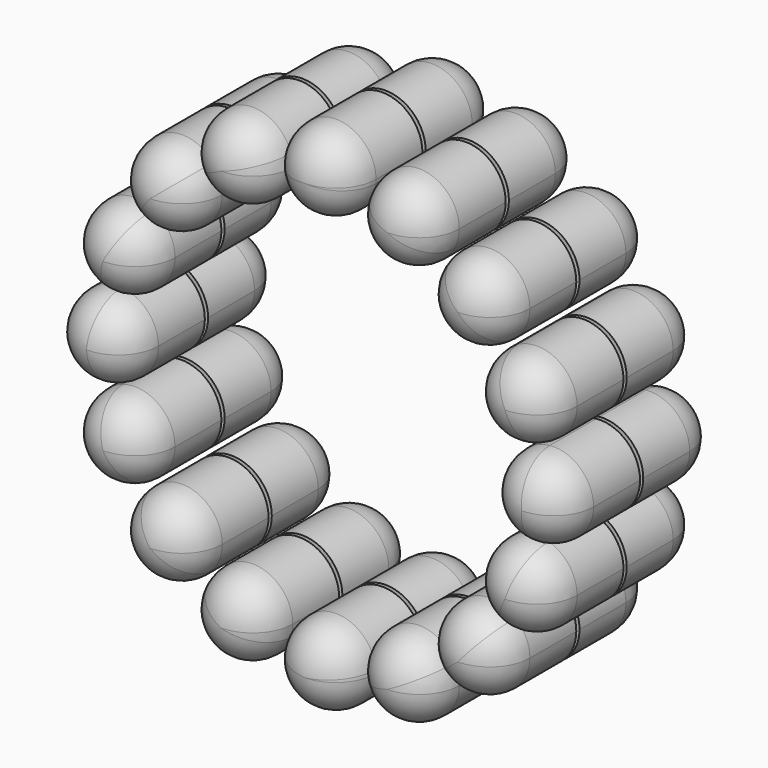
from build123d import *

# Parameters (mm, degrees)
F1_START      = 0.1
F1_DEPTH      = 4.9
F4_START      = -0.1
F4_DEPTH      = 4.9
F5_R          = 2
F5_2_R        = 2
F5_3_R        = 2
F5_4_R        = 2
F5_5_R        = 2
F5_6_R        = 2
F5_7_R        = 2
F5_8_R        = 2
F5_9_R        = 2
F5_10_R       = 2
F5_11_R       = 2
F5_12_R       = 2
F5_13_R       = 2
F5_14_R       = 2
F5_15_R       = 2
F5_16_R       = 2
F5_17_R       = 2
F5_18_R       = 2
F5_19_R       = 2
F5_20_R       = 2
F5_21_R       = 2
F5_22_R       = 2
F5_23_R       = 2
F5_24_R       = 2
F5_25_R       = 2
F5_26_R       = 2
F5_27_R       = 2
F5_28_R       = 2
F5_29_R       = 2
F5_30_R       = 2
F5_31_R       = 2
F5_32_R       = 2
F6_DEPTH      = 0.4
F6_DEPTH_BACK = 0.4


# Not quite as in the source:
# - the program builds the solid bodies; features that only make, move or delete a surface that nothing else refers to are left out


with BuildPart() as f1:
    # F0 (on Front) → F1 (new body)
    with BuildSketch(Plane.XZ.offset(F1_START)):
        with BuildLine():
            ThreePointArc((-1.9915265076, 10.691091954), (0, 8.875), (1.9915265076, 10.691091954))
            ThreePointArc((1.9915265076, 10.691091954), (1.8433395216, 10.717636139), (1.6947992849, 10.7421264368))
            ThreePointArc((1.6947992849, 10.7421264368), (0, 9.175), (-1.6947992849, 10.7421264368))
            ThreePointArc((-1.6947992849, 10.7421264368), (-1.8433395216, 10.717636139), (-1.9915265076, 10.691091954))
        make_face()
        with BuildLine():
            ThreePointArc((1.6947992849, 10.7421264368), (1.8433395216, 10.717636139), (1.9915265076, 10.691091954))
            ThreePointArc((1.9915265076, 10.691091954), (1.9978805038, 10.7829484255), (2, 10.875))
            ThreePointArc((2, 10.875), (-0.0920515745, 12.8728805038), (-1.9915265076, 10.691091954))
            ThreePointArc((-1.9915265076, 10.691091954), (-1.8433395216, 10.717636139), (-1.6947992849, 10.7421264368))
            ThreePointArc((-1.6947992849, 10.7421264368), (-0.0664876516, 12.5736993237), (1.7, 10.875))
            ThreePointArc((1.7, 10.875), (1.6986993237, 10.8085123484), (1.6947992849, 10.7421264368))
        make_face()
        with BuildLine():
            ThreePointArc((-1.6947992849, 10.7421264368), (0, 10.875), (1.6947992849, 10.7421264368))
            ThreePointArc((1.6947992849, 10.7421264368), (1.6986993237, 10.8085123484), (1.7, 10.875))
            ThreePointArc((1.7, 10.875), (-0.0664876516, 12.5736993237), (-1.6947992849, 10.7421264368))
        make_face()
        with BuildLine():
            ThreePointArc((-1.6947992849, 10.7421264368), (0, 9.175), (1.6947992849, 10.7421264368))
            ThreePointArc((1.6947992849, 10.7421264368), (0, 10.875), (-1.6947992849, 10.7421264368))
        make_face()
    extrude(amount=F1_DEPTH)

    # F5#3
    f5_3_edges = [f1.edges().sort_by_distance(p)[0] for p in [
        (-1.991527, -5, 11.058908),
    ]]
    fillet(f5_3_edges, radius=F5_3_R)


with BuildPart() as f1b:
    # F0 (on Front) → F1, piece 2 (new body)
    with BuildSketch(Plane.XZ.offset(F1_START)):
        with BuildLine():
            ThreePointArc((2.2513731858, 10.6394052361), (3.3963154622, 8.199430851), (5.9312343436, 9.1151568369))
            ThreePointArc((5.9312343436, 9.1151568369), (5.80448544, 9.1963891706), (5.6766241868, 9.2758591431))
            ThreePointArc((5.6766241868, 9.2758591431), (3.5111204919, 8.4765947108), (2.5450434447, 10.5730023581))
            ThreePointArc((2.5450434447, 10.5730023581), (2.3984381291, 10.6072201609), (2.2513731858, 10.6394052361))
        make_face()
        with BuildLine():
            ThreePointArc((5.6766241868, 9.2758591431), (5.80448544, 9.1963891706), (5.9312343436, 9.1151568369))
            ThreePointArc((5.9312343436, 9.1151568369), (6.1032157458, 9.5671399359), (6.161682327, 10.0471899161))
            ThreePointArc((6.161682327, 10.0471899161), (4.4611666485, 12.0246400775), (2.2513731858, 10.6394052361))
            ThreePointArc((2.2513731858, 10.6394052361), (2.3984381291, 10.6072201609), (2.5450434447, 10.5730023581))
            ThreePointArc((2.5450434447, 10.5730023581), (4.4278720151, 11.7262203059), (5.861682327, 10.0471899161))
            ThreePointArc((5.861682327, 10.0471899161), (5.8147705221, 9.650580008), (5.6766241868, 9.2758591431))
        make_face()
        with BuildLine():
            ThreePointArc((2.5450434447, 10.5730023581), (4.161682327, 10.0471899161), (5.6766241868, 9.2758591431))
            ThreePointArc((5.6766241868, 9.2758591431), (5.8147705221, 9.650580008), (5.861682327, 10.0471899161))
            ThreePointArc((5.861682327, 10.0471899161), (4.4278720151, 11.7262203059), (2.5450434447, 10.5730023581))
        make_face()
        with BuildLine():
            ThreePointArc((2.5450434447, 10.5730023581), (3.5111204919, 8.4765947108), (5.6766241868, 9.2758591431))
            ThreePointArc((5.6766241868, 9.2758591431), (4.161682327, 10.0471899161), (2.5450434447, 10.5730023581))
        make_face()
    extrude(amount=F1_DEPTH)

    # F5#4
    f5_4_edges = [f1b.edges().sort_by_distance(p)[0] for p in [
        (2.39213, -5, 10.979223),
    ]]
    fillet(f5_4_edges, radius=F5_4_R)


with BuildPart() as f1c:
    # F0 (on Front) → F1, piece 3 (new body)
    with BuildSketch(Plane.XZ.offset(F1_START)):
        with BuildLine():
            ThreePointArc((6.1515217205, 8.9679655174), (6.275572683, 6.275572683), (8.9679655174, 6.1515217205))
            ThreePointArc((8.9679655174, 6.1515217205), (8.8819510679, 6.2750753164), (8.7942345149, 6.3974263807))
            ThreePointArc((8.7942345149, 6.3974263807), (6.4877047174, 6.4877047174), (6.3974263807, 8.7942345149))
            ThreePointArc((6.3974263807, 8.7942345149), (6.2750753164, 8.8819510679), (6.1515217205, 8.9679655174))
        make_face()
        with BuildLine():
            ThreePointArc((8.7942345149, 6.3974263807), (8.8819510679, 6.2750753164), (8.9679655174, 6.1515217205))
            ThreePointArc((8.9679655174, 6.1515217205), (9.5003605388, 6.8401859112), (9.6897862454, 7.6897862454))
            ThreePointArc((9.6897862454, 7.6897862454), (8.3692974485, 9.5708137638), (6.1515217205, 8.9679655174))
            ThreePointArc((6.1515217205, 8.9679655174), (6.2750753164, 8.8819510679), (6.3974263807, 8.7942345149))
            ThreePointArc((6.3974263807, 8.7942345149), (8.2784237527, 9.2846235051), (9.3897862454, 7.6897862454))
            ThreePointArc((9.3897862454, 7.6897862454), (9.2337360597, 6.9782955772), (8.7942345149, 6.3974263807))
        make_face()
        with BuildLine():
            ThreePointArc((6.3974263807, 8.7942345149), (7.6897862454, 7.6897862454), (8.7942345149, 6.3974263807))
            ThreePointArc((8.7942345149, 6.3974263807), (9.2337360597, 6.9782955772), (9.3897862454, 7.6897862454))
            ThreePointArc((9.3897862454, 7.6897862454), (8.2784237527, 9.2846235051), (6.3974263807, 8.7942345149))
        make_face()
        with BuildLine():
            ThreePointArc((6.3974263807, 8.7942345149), (6.4877047174, 6.4877047174), (8.7942345149, 6.3974263807))
            ThreePointArc((8.7942345149, 6.3974263807), (7.6897862454, 7.6897862454), (6.3974263807, 8.7942345149))
        make_face()
    extrude(amount=F1_DEPTH)

    # F5#5
    f5_5_edges = [f1c.edges().sort_by_distance(p)[0] for p in [
        (6.411607, -5, 9.228051),
    ]]
    fillet(f5_5_edges, radius=F5_5_R)


with BuildPart() as f1d:
    # F0 (on Front) → F1, piece 4 (new body)
    with BuildSketch(Plane.XZ.offset(F1_START)):
        with BuildLine():
            ThreePointArc((9.1151568369, 5.9312343436), (8.199430851, 3.3963154622), (10.6394052361, 2.2513731858))
            ThreePointArc((10.6394052361, 2.2513731858), (10.6072201609, 2.3984381291), (10.5730023581, 2.5450434447))
            ThreePointArc((10.5730023581, 2.5450434447), (8.4765947108, 3.5111204919), (9.2758591431, 5.6766241868))
            ThreePointArc((9.2758591431, 5.6766241868), (9.1963891706, 5.80448544), (9.1151568369, 5.9312343436))
        make_face()
        with BuildLine():
            ThreePointArc((10.5730023581, 2.5450434447), (10.6072201609, 2.3984381291), (10.6394052361, 2.2513731858))
            ThreePointArc((10.6394052361, 2.2513731858), (11.6572257293, 2.975181303), (12.0471899161, 4.161682327))
            ThreePointArc((12.0471899161, 4.161682327), (11.0806147662, 5.8740003696), (9.1151568369, 5.9312343436))
            ThreePointArc((9.1151568369, 5.9312343436), (9.1963891706, 5.80448544), (9.2758591431, 5.6766241868))
            ThreePointArc((9.2758591431, 5.6766241868), (10.9356542333, 5.6110377551), (11.7471899161, 4.161682327))
            ThreePointArc((11.7471899161, 4.161682327), (11.422668224, 3.162653086), (10.5730023581, 2.5450434447))
        make_face()
        with BuildLine():
            ThreePointArc((9.2758591431, 5.6766241868), (10.0471899161, 4.161682327), (10.5730023581, 2.5450434447))
            ThreePointArc((10.5730023581, 2.5450434447), (11.422668224, 3.162653086), (11.7471899161, 4.161682327))
            ThreePointArc((11.7471899161, 4.161682327), (10.9356542333, 5.6110377551), (9.2758591431, 5.6766241868))
        make_face()
        with BuildLine():
            ThreePointArc((9.2758591431, 5.6766241868), (8.4765947108, 3.5111204919), (10.5730023581, 2.5450434447))
            ThreePointArc((10.5730023581, 2.5450434447), (10.0471899161, 4.161682327), (9.2758591431, 5.6766241868))
        make_face()
    extrude(amount=F1_DEPTH)

    # F5#6
    f5_6_edges = [f1d.edges().sort_by_distance(p)[0] for p in [
        (9.454975, -5, 6.071991),
    ]]
    fillet(f5_6_edges, radius=F5_6_R)


with BuildPart() as f1e:
    # F0 (on Front) → F1, piece 5 (new body)
    with BuildSketch(Plane.XZ.offset(F1_START)):
        with BuildLine():
            ThreePointArc((10.7421264368, -1.6947992849), (9.175, 0), (10.7421264368, 1.6947992849))
            ThreePointArc((10.7421264368, 1.6947992849), (10.717636139, 1.8433395216), (10.691091954, 1.9915265076))
            ThreePointArc((10.691091954, 1.9915265076), (8.875, 0), (10.691091954, -1.9915265076))
            ThreePointArc((10.691091954, -1.9915265076), (10.717636139, -1.8433395216), (10.7421264368, -1.6947992849))
        make_face()
        with BuildLine():
            ThreePointArc((10.691091954, 1.9915265076), (10.717636139, 1.8433395216), (10.7421264368, 1.6947992849))
            ThreePointArc((10.7421264368, 1.6947992849), (12.0291479417, 1.2481756802), (12.575, 0))
            ThreePointArc((12.575, 0), (12.0291479417, -1.2481756802), (10.7421264368, -1.6947992849))
            ThreePointArc((10.7421264368, -1.6947992849), (10.717636139, -1.8433395216), (10.691091954, -1.9915265076))
            ThreePointArc((10.691091954, -1.9915265076), (12.2226245597, -1.4778051448), (12.875, 0))
            ThreePointArc((12.875, 0), (12.2226245597, 1.4778051448), (10.691091954, 1.9915265076))
        make_face()
        with BuildLine():
            ThreePointArc((10.7421264368, 1.6947992849), (10.8417307198, 0.85), (10.875, 0))
            ThreePointArc((10.875, 0), (10.8417307198, -0.85), (10.7421264368, -1.6947992849))
            ThreePointArc((10.7421264368, -1.6947992849), (12.0291479417, -1.2481756802), (12.575, 0))
            ThreePointArc((12.575, 0), (12.0291479417, 1.2481756802), (10.7421264368, 1.6947992849))
        make_face()
        with BuildLine():
            ThreePointArc((10.7421264368, -1.6947992849), (10.8417307198, -0.85), (10.875, 0))
            ThreePointArc((10.875, 0), (10.8417307198, 0.85), (10.7421264368, 1.6947992849))
            ThreePointArc((10.7421264368, 1.6947992849), (9.175, 0), (10.7421264368, -1.6947992849))
        make_face()
    extrude(amount=F1_DEPTH)

    # F5#7
    f5_7_edges = [f1e.edges().sort_by_distance(p)[0] for p in [
        (11.058908, -5, 1.991527),
    ]]
    fillet(f5_7_edges, radius=F5_7_R)


with BuildPart() as f1f:
    # F0 (on Front) → F1, piece 6 (new body)
    with BuildSketch(Plane.XZ.offset(F1_START)):
        with BuildLine():
            ThreePointArc((10.5730023581, -2.5450434447), (10.6072201609, -2.3984381291), (10.6394052361, -2.2513731858))
            ThreePointArc((10.6394052361, -2.2513731858), (8.199430851, -3.3963154622), (9.1151568369, -5.9312343436))
            ThreePointArc((9.1151568369, -5.9312343436), (9.1963891706, -5.80448544), (9.2758591431, -5.6766241868))
            ThreePointArc((9.2758591431, -5.6766241868), (8.4765947108, -3.5111204919), (10.5730023581, -2.5450434447))
        make_face()
        with BuildLine():
            ThreePointArc((12.0471899161, -4.161682327), (11.6572257293, -2.975181303), (10.6394052361, -2.2513731858))
            ThreePointArc((10.6394052361, -2.2513731858), (10.6072201609, -2.3984381291), (10.5730023581, -2.5450434447))
            ThreePointArc((10.5730023581, -2.5450434447), (11.422668224, -3.162653086), (11.7471899161, -4.161682327))
            ThreePointArc((11.7471899161, -4.161682327), (10.9356542333, -5.6110377551), (9.2758591431, -5.6766241868))
            ThreePointArc((9.2758591431, -5.6766241868), (9.1963891706, -5.80448544), (9.1151568369, -5.9312343436))
            ThreePointArc((9.1151568369, -5.9312343436), (11.0806147662, -5.8740003696), (12.0471899161, -4.161682327))
        make_face()
        with BuildLine():
            ThreePointArc((11.7471899161, -4.161682327), (11.422668224, -3.162653086), (10.5730023581, -2.5450434447))
            ThreePointArc((10.5730023581, -2.5450434447), (10.0471899161, -4.161682327), (9.2758591431, -5.6766241868))
            ThreePointArc((9.2758591431, -5.6766241868), (10.9356542333, -5.6110377551), (11.7471899161, -4.161682327))
        make_face()
        with BuildLine():
            ThreePointArc((9.2758591431, -5.6766241868), (10.0471899161, -4.161682327), (10.5730023581, -2.5450434447))
            ThreePointArc((10.5730023581, -2.5450434447), (8.4765947108, -3.5111204919), (9.2758591431, -5.6766241868))
        make_face()
    extrude(amount=F1_DEPTH)

    # F5#8
    f5_8_edges = [f1f.edges().sort_by_distance(p)[0] for p in [
        (10.979223, -5, -2.39213),
    ]]
    fillet(f5_8_edges, radius=F5_8_R)


with BuildPart() as f1g:
    # F0 (on Front) → F1, piece 7 (new body)
    with BuildSketch(Plane.XZ.offset(F1_START)):
        with BuildLine():
            ThreePointArc((8.7942345149, -6.3974263807), (8.8819510679, -6.2750753164), (8.9679655174, -6.1515217205))
            ThreePointArc((8.9679655174, -6.1515217205), (6.275572683, -6.275572683), (6.1515217205, -8.9679655174))
            ThreePointArc((6.1515217205, -8.9679655174), (6.2750753164, -8.8819510679), (6.3974263807, -8.7942345149))
            ThreePointArc((6.3974263807, -8.7942345149), (6.4877047174, -6.4877047174), (8.7942345149, -6.3974263807))
        make_face()
        with BuildLine():
            ThreePointArc((9.6897862454, -7.6897862454), (9.5003605388, -6.8401859112), (8.9679655174, -6.1515217205))
            ThreePointArc((8.9679655174, -6.1515217205), (8.8819510679, -6.2750753164), (8.7942345149, -6.3974263807))
            ThreePointArc((8.7942345149, -6.3974263807), (9.2337360597, -6.9782955772), (9.3897862454, -7.6897862454))
            ThreePointArc((9.3897862454, -7.6897862454), (8.2784237527, -9.2846235051), (6.3974263807, -8.7942345149))
            ThreePointArc((6.3974263807, -8.7942345149), (6.2750753164, -8.8819510679), (6.1515217205, -8.9679655174))
            ThreePointArc((6.1515217205, -8.9679655174), (8.3692974485, -9.5708137638), (9.6897862454, -7.6897862454))
        make_face()
        with BuildLine():
            ThreePointArc((9.3897862454, -7.6897862454), (9.2337360597, -6.9782955772), (8.7942345149, -6.3974263807))
            ThreePointArc((8.7942345149, -6.3974263807), (7.6897862454, -7.6897862454), (6.3974263807, -8.7942345149))
            ThreePointArc((6.3974263807, -8.7942345149), (8.2784237527, -9.2846235051), (9.3897862454, -7.6897862454))
        make_face()
        with BuildLine():
            ThreePointArc((6.3974263807, -8.7942345149), (7.6897862454, -7.6897862454), (8.7942345149, -6.3974263807))
            ThreePointArc((8.7942345149, -6.3974263807), (6.4877047174, -6.4877047174), (6.3974263807, -8.7942345149))
        make_face()
    extrude(amount=F1_DEPTH)

    # F5#9
    f5_9_edges = [f1g.edges().sort_by_distance(p)[0] for p in [
        (9.228051, -5, -6.411607),
    ]]
    fillet(f5_9_edges, radius=F5_9_R)


with BuildPart() as f1h:
    # F0 (on Front) → F1, piece 8 (new body)
    with BuildSketch(Plane.XZ.offset(F1_START)):
        with BuildLine():
            ThreePointArc((5.6766241868, -9.2758591431), (5.80448544, -9.1963891706), (5.9312343436, -9.1151568369))
            ThreePointArc((5.9312343436, -9.1151568369), (3.3963154622, -8.199430851), (2.2513731858, -10.6394052361))
            ThreePointArc((2.2513731858, -10.6394052361), (2.3984381291, -10.6072201609), (2.5450434447, -10.5730023581))
            ThreePointArc((2.5450434447, -10.5730023581), (3.5111204919, -8.4765947108), (5.6766241868, -9.2758591431))
        make_face()
        with BuildLine():
            ThreePointArc((6.161682327, -10.0471899161), (6.1032157458, -9.5671399359), (5.9312343436, -9.1151568369))
            ThreePointArc((5.9312343436, -9.1151568369), (5.80448544, -9.1963891706), (5.6766241868, -9.2758591431))
            ThreePointArc((5.6766241868, -9.2758591431), (5.8147705221, -9.650580008), (5.861682327, -10.0471899161))
            ThreePointArc((5.861682327, -10.0471899161), (4.4278720151, -11.7262203059), (2.5450434447, -10.5730023581))
            ThreePointArc((2.5450434447, -10.5730023581), (2.3984381291, -10.6072201609), (2.2513731858, -10.6394052361))
            ThreePointArc((2.2513731858, -10.6394052361), (4.4611666485, -12.0246400775), (6.161682327, -10.0471899161))
        make_face()
        with BuildLine():
            ThreePointArc((5.861682327, -10.0471899161), (5.8147705221, -9.650580008), (5.6766241868, -9.2758591431))
            ThreePointArc((5.6766241868, -9.2758591431), (4.161682327, -10.0471899161), (2.5450434447, -10.5730023581))
            ThreePointArc((2.5450434447, -10.5730023581), (4.4278720151, -11.7262203059), (5.861682327, -10.0471899161))
        make_face()
        with BuildLine():
            ThreePointArc((2.5450434447, -10.5730023581), (4.161682327, -10.0471899161), (5.6766241868, -9.2758591431))
            ThreePointArc((5.6766241868, -9.2758591431), (3.5111204919, -8.4765947108), (2.5450434447, -10.5730023581))
        make_face()
    extrude(amount=F1_DEPTH)

    # F5#10
    f5_10_edges = [f1h.edges().sort_by_distance(p)[0] for p in [
        (6.071991, -5, -9.454975),
    ]]
    fillet(f5_10_edges, radius=F5_10_R)


with BuildPart() as f1i:
    # F0 (on Front) → F1, piece 9 (new body)
    with BuildSketch(Plane.XZ.offset(F1_START)):
        with BuildLine():
            ThreePointArc((1.6947992849, -10.7421264368), (1.8433395216, -10.717636139), (1.9915265076, -10.691091954))
            ThreePointArc((1.9915265076, -10.691091954), (0, -8.875), (-1.9915265076, -10.691091954))
            ThreePointArc((-1.9915265076, -10.691091954), (-1.8433395216, -10.717636139), (-1.6947992849, -10.7421264368))
            ThreePointArc((-1.6947992849, -10.7421264368), (0, -9.175), (1.6947992849, -10.7421264368))
        make_face()
        with BuildLine():
            ThreePointArc((2, -10.875), (1.9978805038, -10.7829484255), (1.9915265076, -10.691091954))
            ThreePointArc((1.9915265076, -10.691091954), (1.8433395216, -10.717636139), (1.6947992849, -10.7421264368))
            ThreePointArc((1.6947992849, -10.7421264368), (1.6986993237, -10.8085123484), (1.7, -10.875))
            ThreePointArc((1.7, -10.875), (-0.0664876516, -12.5736993237), (-1.6947992849, -10.7421264368))
            ThreePointArc((-1.6947992849, -10.7421264368), (-1.8433395216, -10.717636139), (-1.9915265076, -10.691091954))
            ThreePointArc((-1.9915265076, -10.691091954), (-0.0920515745, -12.8728805038), (2, -10.875))
        make_face()
        with BuildLine():
            ThreePointArc((1.7, -10.875), (1.6986993237, -10.8085123484), (1.6947992849, -10.7421264368))
            ThreePointArc((1.6947992849, -10.7421264368), (0, -10.875), (-1.6947992849, -10.7421264368))
            ThreePointArc((-1.6947992849, -10.7421264368), (-0.0664876516, -12.5736993237), (1.7, -10.875))
        make_face()
        with BuildLine():
            ThreePointArc((-1.6947992849, -10.7421264368), (0, -10.875), (1.6947992849, -10.7421264368))
            ThreePointArc((1.6947992849, -10.7421264368), (0, -9.175), (-1.6947992849, -10.7421264368))
        make_face()
    extrude(amount=F1_DEPTH)

    # F5#11
    f5_11_edges = [f1i.edges().sort_by_distance(p)[0] for p in [
        (1.991527, -5, -11.058908),
    ]]
    fillet(f5_11_edges, radius=F5_11_R)


with BuildPart() as f1j:
    # F0 (on Front) → F1, piece 10 (new body)
    with BuildSketch(Plane.XZ.offset(F1_START)):
        with BuildLine():
            ThreePointArc((-5.9312343436, -9.1151568369), (-4.9270491917, -11.8949489811), (-2.2513731858, -10.6394052361))
            ThreePointArc((-2.2513731858, -10.6394052361), (-2.3984381291, -10.6072201609), (-2.5450434447, -10.5730023581))
            ThreePointArc((-2.5450434447, -10.5730023581), (-4.812244162, -11.6177851213), (-5.6766241868, -9.2758591431))
            ThreePointArc((-5.6766241868, -9.2758591431), (-5.80448544, -9.1963891706), (-5.9312343436, -9.1151568369))
        make_face()
        with BuildLine():
            ThreePointArc((-2.5450434447, -10.5730023581), (-2.3984381291, -10.6072201609), (-2.2513731858, -10.6394052361))
            ThreePointArc((-2.2513731858, -10.6394052361), (-2.1842321655, -10.3466742376), (-2.161682327, -10.0471899161))
            ThreePointArc((-2.161682327, -10.0471899161), (-3.6816323468, -8.1056564972), (-5.9312343436, -9.1151568369))
            ThreePointArc((-5.9312343436, -9.1151568369), (-5.80448544, -9.1963891706), (-5.6766241868, -9.2758591431))
            ThreePointArc((-5.6766241868, -9.2758591431), (-3.7650724189, -8.3941017209), (-2.461682327, -10.0471899161))
            ThreePointArc((-2.461682327, -10.0471899161), (-2.4826519371, -10.3133796041), (-2.5450434447, -10.5730023581))
        make_face()
        with BuildLine():
            ThreePointArc((-5.6766241868, -9.2758591431), (-4.812244162, -11.6177851213), (-2.5450434447, -10.5730023581))
            ThreePointArc((-2.5450434447, -10.5730023581), (-4.161682327, -10.0471899161), (-5.6766241868, -9.2758591431))
        make_face()
        with BuildLine():
            ThreePointArc((-5.6766241868, -9.2758591431), (-4.161682327, -10.0471899161), (-2.5450434447, -10.5730023581))
            ThreePointArc((-2.5450434447, -10.5730023581), (-2.4826519371, -10.3133796041), (-2.461682327, -10.0471899161))
            ThreePointArc((-2.461682327, -10.0471899161), (-3.7650724189, -8.3941017209), (-5.6766241868, -9.2758591431))
        make_face()
    extrude(amount=F1_DEPTH)

    # F5#12
    f5_12_edges = [f1j.edges().sort_by_distance(p)[0] for p in [
        (-6.071991, -5, -9.454975),
    ]]
    fillet(f5_12_edges, radius=F5_12_R)


with BuildPart() as f1k:
    # F0 (on Front) → F1, piece 11 (new body)
    with BuildSketch(Plane.XZ.offset(F1_START)):
        with BuildLine():
            ThreePointArc((-8.9679655174, -6.1515217205), (-9.1039998078, -9.1039998078), (-6.1515217205, -8.9679655174))
            ThreePointArc((-6.1515217205, -8.9679655174), (-6.2750753164, -8.8819510679), (-6.3974263807, -8.7942345149))
            ThreePointArc((-6.3974263807, -8.7942345149), (-8.8918677734, -8.8918677734), (-8.7942345149, -6.3974263807))
            ThreePointArc((-8.7942345149, -6.3974263807), (-8.8819510679, -6.2750753164), (-8.9679655174, -6.1515217205))
        make_face()
        with BuildLine():
            ThreePointArc((-6.3974263807, -8.7942345149), (-6.2750753164, -8.8819510679), (-6.1515217205, -8.9679655174))
            ThreePointArc((-6.1515217205, -8.9679655174), (-5.808758727, -8.3692974485), (-5.6897862454, -7.6897862454))
            ThreePointArc((-5.6897862454, -7.6897862454), (-6.8401859112, -5.879211952), (-8.9679655174, -6.1515217205))
            ThreePointArc((-8.9679655174, -6.1515217205), (-8.8819510679, -6.2750753164), (-8.7942345149, -6.3974263807))
            ThreePointArc((-8.7942345149, -6.3974263807), (-6.9782955772, -6.1458364311), (-5.9897862454, -7.6897862454))
            ThreePointArc((-5.9897862454, -7.6897862454), (-6.0949489857, -8.2784237527), (-6.3974263807, -8.7942345149))
        make_face()
        with BuildLine():
            ThreePointArc((-8.7942345149, -6.3974263807), (-8.8918677734, -8.8918677734), (-6.3974263807, -8.7942345149))
            ThreePointArc((-6.3974263807, -8.7942345149), (-7.6897862454, -7.6897862454), (-8.7942345149, -6.3974263807))
        make_face()
        with BuildLine():
            ThreePointArc((-8.7942345149, -6.3974263807), (-7.6897862454, -7.6897862454), (-6.3974263807, -8.7942345149))
            ThreePointArc((-6.3974263807, -8.7942345149), (-6.0949489857, -8.2784237527), (-5.9897862454, -7.6897862454))
            ThreePointArc((-5.9897862454, -7.6897862454), (-6.9782955772, -6.1458364311), (-8.7942345149, -6.3974263807))
        make_face()
    extrude(amount=F1_DEPTH)

    # F5#13
    f5_13_edges = [f1k.edges().sort_by_distance(p)[0] for p in [
        (-9.228051, -5, -6.411607),
    ]]
    fillet(f5_13_edges, radius=F5_13_R)


with BuildPart() as f1l:
    # F0 (on Front) → F1, piece 12 (new body)
    with BuildSketch(Plane.XZ.offset(F1_START)):
        with BuildLine():
            ThreePointArc((-10.6394052361, -2.2513731858), (-11.8949489811, -4.9270491917), (-9.1151568369, -5.9312343436))
            ThreePointArc((-9.1151568369, -5.9312343436), (-9.1963891706, -5.80448544), (-9.2758591431, -5.6766241868))
            ThreePointArc((-9.2758591431, -5.6766241868), (-11.6177851213, -4.812244162), (-10.5730023581, -2.5450434447))
            ThreePointArc((-10.5730023581, -2.5450434447), (-10.6072201609, -2.3984381291), (-10.6394052361, -2.2513731858))
        make_face()
        with BuildLine():
            ThreePointArc((-9.2758591431, -5.6766241868), (-9.1963891706, -5.80448544), (-9.1151568369, -5.9312343436))
            ThreePointArc((-9.1151568369, -5.9312343436), (-8.3348718734, -5.1951071771), (-8.0471899161, -4.161682327))
            ThreePointArc((-8.0471899161, -4.161682327), (-8.8606888921, -2.5516465137), (-10.6394052361, -2.2513731858))
            ThreePointArc((-10.6394052361, -2.2513731858), (-10.6072201609, -2.3984381291), (-10.5730023581, -2.5450434447))
            ThreePointArc((-10.5730023581, -2.5450434447), (-9.0481606751, -2.786204019), (-8.3471899161, -4.161682327))
            ThreePointArc((-8.3471899161, -4.161682327), (-8.5978344879, -5.0501466442), (-9.2758591431, -5.6766241868))
        make_face()
        with BuildLine():
            ThreePointArc((-10.5730023581, -2.5450434447), (-11.6177851213, -4.812244162), (-9.2758591431, -5.6766241868))
            ThreePointArc((-9.2758591431, -5.6766241868), (-10.0471899161, -4.161682327), (-10.5730023581, -2.5450434447))
        make_face()
        with BuildLine():
            ThreePointArc((-10.5730023581, -2.5450434447), (-10.0471899161, -4.161682327), (-9.2758591431, -5.6766241868))
            ThreePointArc((-9.2758591431, -5.6766241868), (-8.5978344879, -5.0501466442), (-8.3471899161, -4.161682327))
            ThreePointArc((-8.3471899161, -4.161682327), (-9.0481606751, -2.786204019), (-10.5730023581, -2.5450434447))
        make_face()
    extrude(amount=F1_DEPTH)

    # F5#14
    f5_14_edges = [f1l.edges().sort_by_distance(p)[0] for p in [
        (-10.979223, -5, -2.39213),
    ]]
    fillet(f5_14_edges, radius=F5_14_R)


with BuildPart() as f1m:
    # F0 (on Front) → F1, piece 13 (new body)
    with BuildSketch(Plane.XZ.offset(F1_START)):
        with BuildLine():
            ThreePointArc((-10.7421264368, 1.6947992849), (-10.717636139, 1.8433395216), (-10.691091954, 1.9915265076))
            ThreePointArc((-10.691091954, 1.9915265076), (-12.875, 0), (-10.691091954, -1.9915265076))
            ThreePointArc((-10.691091954, -1.9915265076), (-10.717636139, -1.8433395216), (-10.7421264368, -1.6947992849))
            ThreePointArc((-10.7421264368, -1.6947992849), (-12.575, 0), (-10.7421264368, 1.6947992849))
        make_face()
        with BuildLine():
            ThreePointArc((-8.875, 0), (-9.3971948552, 1.3476245597), (-10.691091954, 1.9915265076))
            ThreePointArc((-10.691091954, 1.9915265076), (-10.717636139, 1.8433395216), (-10.7421264368, 1.6947992849))
            ThreePointArc((-10.7421264368, 1.6947992849), (-9.6268243198, 1.1541479417), (-9.175, 0))
            ThreePointArc((-9.175, 0), (-9.6268243198, -1.1541479417), (-10.7421264368, -1.6947992849))
            ThreePointArc((-10.7421264368, -1.6947992849), (-10.717636139, -1.8433395216), (-10.691091954, -1.9915265076))
            ThreePointArc((-10.691091954, -1.9915265076), (-9.3971948552, -1.3476245597), (-8.875, 0))
        make_face()
        with BuildLine():
            ThreePointArc((-10.7421264368, -1.6947992849), (-10.875, 0), (-10.7421264368, 1.6947992849))
            ThreePointArc((-10.7421264368, 1.6947992849), (-12.575, 0), (-10.7421264368, -1.6947992849))
        make_face()
        with BuildLine():
            ThreePointArc((-9.175, 0), (-9.6268243198, 1.1541479417), (-10.7421264368, 1.6947992849))
            ThreePointArc((-10.7421264368, 1.6947992849), (-10.875, 0), (-10.7421264368, -1.6947992849))
            ThreePointArc((-10.7421264368, -1.6947992849), (-9.6268243198, -1.1541479417), (-9.175, 0))
        make_face()
    extrude(amount=F1_DEPTH)

    # F5#15
    f5_15_edges = [f1m.edges().sort_by_distance(p)[0] for p in [
        (-11.058908, -5, 1.991527),
    ]]
    fillet(f5_15_edges, radius=F5_15_R)


with BuildPart() as f1n:
    # F0 (on Front) → F1, piece 14 (new body)
    with BuildSketch(Plane.XZ.offset(F1_START)):
        with BuildLine():
            ThreePointArc((-9.2758591431, 5.6766241868), (-9.1963891706, 5.80448544), (-9.1151568369, 5.9312343436))
            ThreePointArc((-9.1151568369, 5.9312343436), (-11.8949489811, 4.9270491917), (-10.6394052361, 2.2513731858))
            ThreePointArc((-10.6394052361, 2.2513731858), (-10.6072201609, 2.3984381291), (-10.5730023581, 2.5450434447))
            ThreePointArc((-10.5730023581, 2.5450434447), (-11.6177851213, 4.812244162), (-9.2758591431, 5.6766241868))
        make_face()
        with BuildLine():
            ThreePointArc((-8.0471899161, 4.161682327), (-8.3348718734, 5.1951071771), (-9.1151568369, 5.9312343436))
            ThreePointArc((-9.1151568369, 5.9312343436), (-9.1963891706, 5.80448544), (-9.2758591431, 5.6766241868))
            ThreePointArc((-9.2758591431, 5.6766241868), (-8.5978344879, 5.0501466442), (-8.3471899161, 4.161682327))
            ThreePointArc((-8.3471899161, 4.161682327), (-9.0481606751, 2.786204019), (-10.5730023581, 2.5450434447))
            ThreePointArc((-10.5730023581, 2.5450434447), (-10.6072201609, 2.3984381291), (-10.6394052361, 2.2513731858))
            ThreePointArc((-10.6394052361, 2.2513731858), (-8.8606888921, 2.5516465137), (-8.0471899161, 4.161682327))
        make_face()
        with BuildLine():
            ThreePointArc((-10.5730023581, 2.5450434447), (-10.0471899161, 4.161682327), (-9.2758591431, 5.6766241868))
            ThreePointArc((-9.2758591431, 5.6766241868), (-11.6177851213, 4.812244162), (-10.5730023581, 2.5450434447))
        make_face()
        with BuildLine():
            ThreePointArc((-8.3471899161, 4.161682327), (-8.5978344879, 5.0501466442), (-9.2758591431, 5.6766241868))
            ThreePointArc((-9.2758591431, 5.6766241868), (-10.0471899161, 4.161682327), (-10.5730023581, 2.5450434447))
            ThreePointArc((-10.5730023581, 2.5450434447), (-9.0481606751, 2.786204019), (-8.3471899161, 4.161682327))
        make_face()
    extrude(amount=F1_DEPTH)

    # F5#16
    f5_16_edges = [f1n.edges().sort_by_distance(p)[0] for p in [
        (-9.454975, -5, 6.071991),
    ]]
    fillet(f5_16_edges, radius=F5_16_R)


with BuildPart() as f1o:
    # F0 (on Front) → F1, piece 15 (new body)
    with BuildSketch(Plane.XZ.offset(F1_START)):
        with BuildLine():
            ThreePointArc((-6.3974263807, 8.7942345149), (-6.2750753164, 8.8819510679), (-6.1515217205, 8.9679655174))
            ThreePointArc((-6.1515217205, 8.9679655174), (-9.1039998078, 9.1039998078), (-8.9679655174, 6.1515217205))
            ThreePointArc((-8.9679655174, 6.1515217205), (-8.8819510679, 6.2750753164), (-8.7942345149, 6.3974263807))
            ThreePointArc((-8.7942345149, 6.3974263807), (-8.8918677734, 8.8918677734), (-6.3974263807, 8.7942345149))
        make_face()
        with BuildLine():
            ThreePointArc((-5.6897862454, 7.6897862454), (-5.808758727, 8.3692974485), (-6.1515217205, 8.9679655174))
            ThreePointArc((-6.1515217205, 8.9679655174), (-6.2750753164, 8.8819510679), (-6.3974263807, 8.7942345149))
            ThreePointArc((-6.3974263807, 8.7942345149), (-6.0949489857, 8.2784237527), (-5.9897862454, 7.6897862454))
            ThreePointArc((-5.9897862454, 7.6897862454), (-6.9782955772, 6.1458364311), (-8.7942345149, 6.3974263807))
            ThreePointArc((-8.7942345149, 6.3974263807), (-8.8819510679, 6.2750753164), (-8.9679655174, 6.1515217205))
            ThreePointArc((-8.9679655174, 6.1515217205), (-6.8401859112, 5.879211952), (-5.6897862454, 7.6897862454))
        make_face()
        with BuildLine():
            ThreePointArc((-8.7942345149, 6.3974263807), (-7.6897862454, 7.6897862454), (-6.3974263807, 8.7942345149))
            ThreePointArc((-6.3974263807, 8.7942345149), (-8.8918677734, 8.8918677734), (-8.7942345149, 6.3974263807))
        make_face()
        with BuildLine():
            ThreePointArc((-5.9897862454, 7.6897862454), (-6.0949489857, 8.2784237527), (-6.3974263807, 8.7942345149))
            ThreePointArc((-6.3974263807, 8.7942345149), (-7.6897862454, 7.6897862454), (-8.7942345149, 6.3974263807))
            ThreePointArc((-8.7942345149, 6.3974263807), (-6.9782955772, 6.1458364311), (-5.9897862454, 7.6897862454))
        make_face()
    extrude(amount=F1_DEPTH)

    # F5
    f5_edges = [f1o.edges().sort_by_distance(p)[0] for p in [
        (-6.411607, -5, 9.228051),
    ]]
    fillet(f5_edges, radius=F5_R)


with BuildPart() as f1p:
    # F0 (on Front) → F1, piece 16 (new body)
    with BuildSketch(Plane.XZ.offset(F1_START)):
        with BuildLine():
            ThreePointArc((-2.5450434447, 10.5730023581), (-2.3984381291, 10.6072201609), (-2.2513731858, 10.6394052361))
            ThreePointArc((-2.2513731858, 10.6394052361), (-4.9270491917, 11.8949489811), (-5.9312343436, 9.1151568369))
            ThreePointArc((-5.9312343436, 9.1151568369), (-5.80448544, 9.1963891706), (-5.6766241868, 9.2758591431))
            ThreePointArc((-5.6766241868, 9.2758591431), (-4.812244162, 11.6177851213), (-2.5450434447, 10.5730023581))
        make_face()
        with BuildLine():
            ThreePointArc((-2.161682327, 10.0471899161), (-2.1842321655, 10.3466742376), (-2.2513731858, 10.6394052361))
            ThreePointArc((-2.2513731858, 10.6394052361), (-2.3984381291, 10.6072201609), (-2.5450434447, 10.5730023581))
            ThreePointArc((-2.5450434447, 10.5730023581), (-2.4826519371, 10.3133796041), (-2.461682327, 10.0471899161))
            ThreePointArc((-2.461682327, 10.0471899161), (-3.7650724189, 8.3941017209), (-5.6766241868, 9.2758591431))
            ThreePointArc((-5.6766241868, 9.2758591431), (-5.80448544, 9.1963891706), (-5.9312343436, 9.1151568369))
            ThreePointArc((-5.9312343436, 9.1151568369), (-3.6816323468, 8.1056564972), (-2.161682327, 10.0471899161))
        make_face()
        with BuildLine():
            ThreePointArc((-5.6766241868, 9.2758591431), (-4.161682327, 10.0471899161), (-2.5450434447, 10.5730023581))
            ThreePointArc((-2.5450434447, 10.5730023581), (-4.812244162, 11.6177851213), (-5.6766241868, 9.2758591431))
        make_face()
        with BuildLine():
            ThreePointArc((-2.461682327, 10.0471899161), (-2.4826519371, 10.3133796041), (-2.5450434447, 10.5730023581))
            ThreePointArc((-2.5450434447, 10.5730023581), (-4.161682327, 10.0471899161), (-5.6766241868, 9.2758591431))
            ThreePointArc((-5.6766241868, 9.2758591431), (-3.7650724189, 8.3941017209), (-2.461682327, 10.0471899161))
        make_face()
    extrude(amount=F1_DEPTH)

    # F5#2
    f5_2_edges = [f1p.edges().sort_by_distance(p)[0] for p in [
        (-2.39213, -5, 10.979223),
    ]]
    fillet(f5_2_edges, radius=F5_2_R)


with BuildPart() as f4:
    # F0 (on Front) → F4 (new body)
    with BuildSketch(Plane.XZ.offset(F4_START)):
        with BuildLine():
            ThreePointArc((11.7471899161, -4.161682327), (11.422668224, -3.162653086), (10.5730023581, -2.5450434447))
            ThreePointArc((10.5730023581, -2.5450434447), (10.0471899161, -4.161682327), (9.2758591431, -5.6766241868))
            ThreePointArc((9.2758591431, -5.6766241868), (10.9356542333, -5.6110377551), (11.7471899161, -4.161682327))
        make_face()
        with BuildLine():
            ThreePointArc((12.0471899161, -4.161682327), (11.6572257293, -2.975181303), (10.6394052361, -2.2513731858))
            ThreePointArc((10.6394052361, -2.2513731858), (10.6072201609, -2.3984381291), (10.5730023581, -2.5450434447))
            ThreePointArc((10.5730023581, -2.5450434447), (11.422668224, -3.162653086), (11.7471899161, -4.161682327))
            ThreePointArc((11.7471899161, -4.161682327), (10.9356542333, -5.6110377551), (9.2758591431, -5.6766241868))
            ThreePointArc((9.2758591431, -5.6766241868), (9.1963891706, -5.80448544), (9.1151568369, -5.9312343436))
            ThreePointArc((9.1151568369, -5.9312343436), (11.0806147662, -5.8740003696), (12.0471899161, -4.161682327))
        make_face()
        with BuildLine():
            ThreePointArc((9.2758591431, -5.6766241868), (10.0471899161, -4.161682327), (10.5730023581, -2.5450434447))
            ThreePointArc((10.5730023581, -2.5450434447), (8.4765947108, -3.5111204919), (9.2758591431, -5.6766241868))
        make_face()
        with BuildLine():
            ThreePointArc((10.5730023581, -2.5450434447), (10.6072201609, -2.3984381291), (10.6394052361, -2.2513731858))
            ThreePointArc((10.6394052361, -2.2513731858), (8.199430851, -3.3963154622), (9.1151568369, -5.9312343436))
            ThreePointArc((9.1151568369, -5.9312343436), (9.1963891706, -5.80448544), (9.2758591431, -5.6766241868))
            ThreePointArc((9.2758591431, -5.6766241868), (8.4765947108, -3.5111204919), (10.5730023581, -2.5450434447))
        make_face()
    extrude(amount=-F4_DEPTH)

    # F5#29
    f5_29_edges = [f4.edges().sort_by_distance(p)[0] for p in [
        (9.454975, 5, -6.071991),
    ]]
    fillet(f5_29_edges, radius=F5_29_R)


with BuildPart() as f4b:
    # F0 (on Front) → F4, piece 2 (new body)
    with BuildSketch(Plane.XZ.offset(F4_START)):
        with BuildLine():
            ThreePointArc((8.7942345149, -6.3974263807), (8.8819510679, -6.2750753164), (8.9679655174, -6.1515217205))
            ThreePointArc((8.9679655174, -6.1515217205), (6.275572683, -6.275572683), (6.1515217205, -8.9679655174))
            ThreePointArc((6.1515217205, -8.9679655174), (6.2750753164, -8.8819510679), (6.3974263807, -8.7942345149))
            ThreePointArc((6.3974263807, -8.7942345149), (6.4877047174, -6.4877047174), (8.7942345149, -6.3974263807))
        make_face()
        with BuildLine():
            ThreePointArc((6.3974263807, -8.7942345149), (7.6897862454, -7.6897862454), (8.7942345149, -6.3974263807))
            ThreePointArc((8.7942345149, -6.3974263807), (6.4877047174, -6.4877047174), (6.3974263807, -8.7942345149))
        make_face()
        with BuildLine():
            ThreePointArc((9.3897862454, -7.6897862454), (9.2337360597, -6.9782955772), (8.7942345149, -6.3974263807))
            ThreePointArc((8.7942345149, -6.3974263807), (7.6897862454, -7.6897862454), (6.3974263807, -8.7942345149))
            ThreePointArc((6.3974263807, -8.7942345149), (8.2784237527, -9.2846235051), (9.3897862454, -7.6897862454))
        make_face()
        with BuildLine():
            ThreePointArc((9.6897862454, -7.6897862454), (9.5003605388, -6.8401859112), (8.9679655174, -6.1515217205))
            ThreePointArc((8.9679655174, -6.1515217205), (8.8819510679, -6.2750753164), (8.7942345149, -6.3974263807))
            ThreePointArc((8.7942345149, -6.3974263807), (9.2337360597, -6.9782955772), (9.3897862454, -7.6897862454))
            ThreePointArc((9.3897862454, -7.6897862454), (8.2784237527, -9.2846235051), (6.3974263807, -8.7942345149))
            ThreePointArc((6.3974263807, -8.7942345149), (6.2750753164, -8.8819510679), (6.1515217205, -8.9679655174))
            ThreePointArc((6.1515217205, -8.9679655174), (8.3692974485, -9.5708137638), (9.6897862454, -7.6897862454))
        make_face()
    extrude(amount=-F4_DEPTH)

    # F5#28
    f5_28_edges = [f4b.edges().sort_by_distance(p)[0] for p in [
        (9.228051, 5, -6.411607),
    ]]
    fillet(f5_28_edges, radius=F5_28_R)


with BuildPart() as f4c:
    # F0 (on Front) → F4, piece 3 (new body)
    with BuildSketch(Plane.XZ.offset(F4_START)):
        with BuildLine():
            ThreePointArc((6.161682327, -10.0471899161), (6.1032157458, -9.5671399359), (5.9312343436, -9.1151568369))
            ThreePointArc((5.9312343436, -9.1151568369), (5.80448544, -9.1963891706), (5.6766241868, -9.2758591431))
            ThreePointArc((5.6766241868, -9.2758591431), (5.8147705221, -9.650580008), (5.861682327, -10.0471899161))
            ThreePointArc((5.861682327, -10.0471899161), (4.4278720151, -11.7262203059), (2.5450434447, -10.5730023581))
            ThreePointArc((2.5450434447, -10.5730023581), (2.3984381291, -10.6072201609), (2.2513731858, -10.6394052361))
            ThreePointArc((2.2513731858, -10.6394052361), (4.4611666485, -12.0246400775), (6.161682327, -10.0471899161))
        make_face()
        with BuildLine():
            ThreePointArc((5.861682327, -10.0471899161), (5.8147705221, -9.650580008), (5.6766241868, -9.2758591431))
            ThreePointArc((5.6766241868, -9.2758591431), (4.161682327, -10.0471899161), (2.5450434447, -10.5730023581))
            ThreePointArc((2.5450434447, -10.5730023581), (4.4278720151, -11.7262203059), (5.861682327, -10.0471899161))
        make_face()
        with BuildLine():
            ThreePointArc((2.5450434447, -10.5730023581), (4.161682327, -10.0471899161), (5.6766241868, -9.2758591431))
            ThreePointArc((5.6766241868, -9.2758591431), (3.5111204919, -8.4765947108), (2.5450434447, -10.5730023581))
        make_face()
        with BuildLine():
            ThreePointArc((5.6766241868, -9.2758591431), (5.80448544, -9.1963891706), (5.9312343436, -9.1151568369))
            ThreePointArc((5.9312343436, -9.1151568369), (3.3963154622, -8.199430851), (2.2513731858, -10.6394052361))
            ThreePointArc((2.2513731858, -10.6394052361), (2.3984381291, -10.6072201609), (2.5450434447, -10.5730023581))
            ThreePointArc((2.5450434447, -10.5730023581), (3.5111204919, -8.4765947108), (5.6766241868, -9.2758591431))
        make_face()
    extrude(amount=-F4_DEPTH)

    # F5#27
    f5_27_edges = [f4c.edges().sort_by_distance(p)[0] for p in [
        (2.39213, 5, -10.979223),
    ]]
    fillet(f5_27_edges, radius=F5_27_R)


with BuildPart() as f4d:
    # F0 (on Front) → F4, piece 4 (new body)
    with BuildSketch(Plane.XZ.offset(F4_START)):
        with BuildLine():
            ThreePointArc((-1.6947992849, -10.7421264368), (0, -10.875), (1.6947992849, -10.7421264368))
            ThreePointArc((1.6947992849, -10.7421264368), (0, -9.175), (-1.6947992849, -10.7421264368))
        make_face()
        with BuildLine():
            ThreePointArc((1.7, -10.875), (1.6986993237, -10.8085123484), (1.6947992849, -10.7421264368))
            ThreePointArc((1.6947992849, -10.7421264368), (0, -10.875), (-1.6947992849, -10.7421264368))
            ThreePointArc((-1.6947992849, -10.7421264368), (-0.0664876516, -12.5736993237), (1.7, -10.875))
        make_face()
        with BuildLine():
            ThreePointArc((2, -10.875), (1.9978805038, -10.7829484255), (1.9915265076, -10.691091954))
            ThreePointArc((1.9915265076, -10.691091954), (1.8433395216, -10.717636139), (1.6947992849, -10.7421264368))
            ThreePointArc((1.6947992849, -10.7421264368), (1.6986993237, -10.8085123484), (1.7, -10.875))
            ThreePointArc((1.7, -10.875), (-0.0664876516, -12.5736993237), (-1.6947992849, -10.7421264368))
            ThreePointArc((-1.6947992849, -10.7421264368), (-1.8433395216, -10.717636139), (-1.9915265076, -10.691091954))
            ThreePointArc((-1.9915265076, -10.691091954), (-0.0920515745, -12.8728805038), (2, -10.875))
        make_face()
        with BuildLine():
            ThreePointArc((1.6947992849, -10.7421264368), (1.8433395216, -10.717636139), (1.9915265076, -10.691091954))
            ThreePointArc((1.9915265076, -10.691091954), (0, -8.875), (-1.9915265076, -10.691091954))
            ThreePointArc((-1.9915265076, -10.691091954), (-1.8433395216, -10.717636139), (-1.6947992849, -10.7421264368))
            ThreePointArc((-1.6947992849, -10.7421264368), (0, -9.175), (1.6947992849, -10.7421264368))
        make_face()
    extrude(amount=-F4_DEPTH)

    # F5#26
    f5_26_edges = [f4d.edges().sort_by_distance(p)[0] for p in [
        (-1.991527, 5, -11.058908),
    ]]
    fillet(f5_26_edges, radius=F5_26_R)


with BuildPart() as f4e:
    # F0 (on Front) → F4, piece 5 (new body)
    with BuildSketch(Plane.XZ.offset(F4_START)):
        with BuildLine():
            ThreePointArc((-2.5450434447, -10.5730023581), (-2.3984381291, -10.6072201609), (-2.2513731858, -10.6394052361))
            ThreePointArc((-2.2513731858, -10.6394052361), (-2.1842321655, -10.3466742376), (-2.161682327, -10.0471899161))
            ThreePointArc((-2.161682327, -10.0471899161), (-3.6816323468, -8.1056564972), (-5.9312343436, -9.1151568369))
            ThreePointArc((-5.9312343436, -9.1151568369), (-5.80448544, -9.1963891706), (-5.6766241868, -9.2758591431))
            ThreePointArc((-5.6766241868, -9.2758591431), (-3.7650724189, -8.3941017209), (-2.461682327, -10.0471899161))
            ThreePointArc((-2.461682327, -10.0471899161), (-2.4826519371, -10.3133796041), (-2.5450434447, -10.5730023581))
        make_face()
        with BuildLine():
            ThreePointArc((-5.6766241868, -9.2758591431), (-4.161682327, -10.0471899161), (-2.5450434447, -10.5730023581))
            ThreePointArc((-2.5450434447, -10.5730023581), (-2.4826519371, -10.3133796041), (-2.461682327, -10.0471899161))
            ThreePointArc((-2.461682327, -10.0471899161), (-3.7650724189, -8.3941017209), (-5.6766241868, -9.2758591431))
        make_face()
        with BuildLine():
            ThreePointArc((-5.6766241868, -9.2758591431), (-4.812244162, -11.6177851213), (-2.5450434447, -10.5730023581))
            ThreePointArc((-2.5450434447, -10.5730023581), (-4.161682327, -10.0471899161), (-5.6766241868, -9.2758591431))
        make_face()
        with BuildLine():
            ThreePointArc((-5.9312343436, -9.1151568369), (-4.9270491917, -11.8949489811), (-2.2513731858, -10.6394052361))
            ThreePointArc((-2.2513731858, -10.6394052361), (-2.3984381291, -10.6072201609), (-2.5450434447, -10.5730023581))
            ThreePointArc((-2.5450434447, -10.5730023581), (-4.812244162, -11.6177851213), (-5.6766241868, -9.2758591431))
            ThreePointArc((-5.6766241868, -9.2758591431), (-5.80448544, -9.1963891706), (-5.9312343436, -9.1151568369))
        make_face()
    extrude(amount=-F4_DEPTH)

    # F5#25
    f5_25_edges = [f4e.edges().sort_by_distance(p)[0] for p in [
        (-2.39213, 5, -10.979223),
    ]]
    fillet(f5_25_edges, radius=F5_25_R)


with BuildPart() as f4f:
    # F0 (on Front) → F4, piece 6 (new body)
    with BuildSketch(Plane.XZ.offset(F4_START)):
        with BuildLine():
            ThreePointArc((-8.9679655174, -6.1515217205), (-9.1039998078, -9.1039998078), (-6.1515217205, -8.9679655174))
            ThreePointArc((-6.1515217205, -8.9679655174), (-6.2750753164, -8.8819510679), (-6.3974263807, -8.7942345149))
            ThreePointArc((-6.3974263807, -8.7942345149), (-8.8918677734, -8.8918677734), (-8.7942345149, -6.3974263807))
            ThreePointArc((-8.7942345149, -6.3974263807), (-8.8819510679, -6.2750753164), (-8.9679655174, -6.1515217205))
        make_face()
        with BuildLine():
            ThreePointArc((-8.7942345149, -6.3974263807), (-8.8918677734, -8.8918677734), (-6.3974263807, -8.7942345149))
            ThreePointArc((-6.3974263807, -8.7942345149), (-7.6897862454, -7.6897862454), (-8.7942345149, -6.3974263807))
        make_face()
        with BuildLine():
            ThreePointArc((-8.7942345149, -6.3974263807), (-7.6897862454, -7.6897862454), (-6.3974263807, -8.7942345149))
            ThreePointArc((-6.3974263807, -8.7942345149), (-6.0949489857, -8.2784237527), (-5.9897862454, -7.6897862454))
            ThreePointArc((-5.9897862454, -7.6897862454), (-6.9782955772, -6.1458364311), (-8.7942345149, -6.3974263807))
        make_face()
        with BuildLine():
            ThreePointArc((-6.3974263807, -8.7942345149), (-6.2750753164, -8.8819510679), (-6.1515217205, -8.9679655174))
            ThreePointArc((-6.1515217205, -8.9679655174), (-5.808758727, -8.3692974485), (-5.6897862454, -7.6897862454))
            ThreePointArc((-5.6897862454, -7.6897862454), (-6.8401859112, -5.879211952), (-8.9679655174, -6.1515217205))
            ThreePointArc((-8.9679655174, -6.1515217205), (-8.8819510679, -6.2750753164), (-8.7942345149, -6.3974263807))
            ThreePointArc((-8.7942345149, -6.3974263807), (-6.9782955772, -6.1458364311), (-5.9897862454, -7.6897862454))
            ThreePointArc((-5.9897862454, -7.6897862454), (-6.0949489857, -8.2784237527), (-6.3974263807, -8.7942345149))
        make_face()
    extrude(amount=-F4_DEPTH)

    # F5#24
    f5_24_edges = [f4f.edges().sort_by_distance(p)[0] for p in [
        (-9.228051, 5, -6.411607),
    ]]
    fillet(f5_24_edges, radius=F5_24_R)


with BuildPart() as f4g:
    # F0 (on Front) → F4, piece 7 (new body)
    with BuildSketch(Plane.XZ.offset(F4_START)):
        with BuildLine():
            ThreePointArc((-10.5730023581, -2.5450434447), (-10.0471899161, -4.161682327), (-9.2758591431, -5.6766241868))
            ThreePointArc((-9.2758591431, -5.6766241868), (-8.5978344879, -5.0501466442), (-8.3471899161, -4.161682327))
            ThreePointArc((-8.3471899161, -4.161682327), (-9.0481606751, -2.786204019), (-10.5730023581, -2.5450434447))
        make_face()
        with BuildLine():
            ThreePointArc((-9.2758591431, -5.6766241868), (-9.1963891706, -5.80448544), (-9.1151568369, -5.9312343436))
            ThreePointArc((-9.1151568369, -5.9312343436), (-8.3348718734, -5.1951071771), (-8.0471899161, -4.161682327))
            ThreePointArc((-8.0471899161, -4.161682327), (-8.8606888921, -2.5516465137), (-10.6394052361, -2.2513731858))
            ThreePointArc((-10.6394052361, -2.2513731858), (-10.6072201609, -2.3984381291), (-10.5730023581, -2.5450434447))
            ThreePointArc((-10.5730023581, -2.5450434447), (-9.0481606751, -2.786204019), (-8.3471899161, -4.161682327))
            ThreePointArc((-8.3471899161, -4.161682327), (-8.5978344879, -5.0501466442), (-9.2758591431, -5.6766241868))
        make_face()
        with BuildLine():
            ThreePointArc((-10.5730023581, -2.5450434447), (-11.6177851213, -4.812244162), (-9.2758591431, -5.6766241868))
            ThreePointArc((-9.2758591431, -5.6766241868), (-10.0471899161, -4.161682327), (-10.5730023581, -2.5450434447))
        make_face()
        with BuildLine():
            ThreePointArc((-10.6394052361, -2.2513731858), (-11.8949489811, -4.9270491917), (-9.1151568369, -5.9312343436))
            ThreePointArc((-9.1151568369, -5.9312343436), (-9.1963891706, -5.80448544), (-9.2758591431, -5.6766241868))
            ThreePointArc((-9.2758591431, -5.6766241868), (-11.6177851213, -4.812244162), (-10.5730023581, -2.5450434447))
            ThreePointArc((-10.5730023581, -2.5450434447), (-10.6072201609, -2.3984381291), (-10.6394052361, -2.2513731858))
        make_face()
    extrude(amount=-F4_DEPTH)

    # F5#23
    f5_23_edges = [f4g.edges().sort_by_distance(p)[0] for p in [
        (-9.454975, 5, -6.071991),
    ]]
    fillet(f5_23_edges, radius=F5_23_R)


with BuildPart() as f4h:
    # F0 (on Front) → F4, piece 8 (new body)
    with BuildSketch(Plane.XZ.offset(F4_START)):
        with BuildLine():
            ThreePointArc((-10.7421264368, 1.6947992849), (-10.717636139, 1.8433395216), (-10.691091954, 1.9915265076))
            ThreePointArc((-10.691091954, 1.9915265076), (-12.875, 0), (-10.691091954, -1.9915265076))
            ThreePointArc((-10.691091954, -1.9915265076), (-10.717636139, -1.8433395216), (-10.7421264368, -1.6947992849))
            ThreePointArc((-10.7421264368, -1.6947992849), (-12.575, 0), (-10.7421264368, 1.6947992849))
        make_face()
        with BuildLine():
            ThreePointArc((-10.7421264368, -1.6947992849), (-10.875, 0), (-10.7421264368, 1.6947992849))
            ThreePointArc((-10.7421264368, 1.6947992849), (-12.575, 0), (-10.7421264368, -1.6947992849))
        make_face()
        with BuildLine():
            ThreePointArc((-9.175, 0), (-9.6268243198, 1.1541479417), (-10.7421264368, 1.6947992849))
            ThreePointArc((-10.7421264368, 1.6947992849), (-10.875, 0), (-10.7421264368, -1.6947992849))
            ThreePointArc((-10.7421264368, -1.6947992849), (-9.6268243198, -1.1541479417), (-9.175, 0))
        make_face()
        with BuildLine():
            ThreePointArc((-8.875, 0), (-9.3971948552, 1.3476245597), (-10.691091954, 1.9915265076))
            ThreePointArc((-10.691091954, 1.9915265076), (-10.717636139, 1.8433395216), (-10.7421264368, 1.6947992849))
            ThreePointArc((-10.7421264368, 1.6947992849), (-9.6268243198, 1.1541479417), (-9.175, 0))
            ThreePointArc((-9.175, 0), (-9.6268243198, -1.1541479417), (-10.7421264368, -1.6947992849))
            ThreePointArc((-10.7421264368, -1.6947992849), (-10.717636139, -1.8433395216), (-10.691091954, -1.9915265076))
            ThreePointArc((-10.691091954, -1.9915265076), (-9.3971948552, -1.3476245597), (-8.875, 0))
        make_face()
    extrude(amount=-F4_DEPTH)

    # F5#22
    f5_22_edges = [f4h.edges().sort_by_distance(p)[0] for p in [
        (-11.058908, 5, 1.991527),
    ]]
    fillet(f5_22_edges, radius=F5_22_R)


with BuildPart() as f4i:
    # F0 (on Front) → F4, piece 9 (new body)
    with BuildSketch(Plane.XZ.offset(F4_START)):
        with BuildLine():
            ThreePointArc((-8.0471899161, 4.161682327), (-8.3348718734, 5.1951071771), (-9.1151568369, 5.9312343436))
            ThreePointArc((-9.1151568369, 5.9312343436), (-9.1963891706, 5.80448544), (-9.2758591431, 5.6766241868))
            ThreePointArc((-9.2758591431, 5.6766241868), (-8.5978344879, 5.0501466442), (-8.3471899161, 4.161682327))
            ThreePointArc((-8.3471899161, 4.161682327), (-9.0481606751, 2.786204019), (-10.5730023581, 2.5450434447))
            ThreePointArc((-10.5730023581, 2.5450434447), (-10.6072201609, 2.3984381291), (-10.6394052361, 2.2513731858))
            ThreePointArc((-10.6394052361, 2.2513731858), (-8.8606888921, 2.5516465137), (-8.0471899161, 4.161682327))
        make_face()
        with BuildLine():
            ThreePointArc((-8.3471899161, 4.161682327), (-8.5978344879, 5.0501466442), (-9.2758591431, 5.6766241868))
            ThreePointArc((-9.2758591431, 5.6766241868), (-10.0471899161, 4.161682327), (-10.5730023581, 2.5450434447))
            ThreePointArc((-10.5730023581, 2.5450434447), (-9.0481606751, 2.786204019), (-8.3471899161, 4.161682327))
        make_face()
        with BuildLine():
            ThreePointArc((-10.5730023581, 2.5450434447), (-10.0471899161, 4.161682327), (-9.2758591431, 5.6766241868))
            ThreePointArc((-9.2758591431, 5.6766241868), (-11.6177851213, 4.812244162), (-10.5730023581, 2.5450434447))
        make_face()
        with BuildLine():
            ThreePointArc((-9.2758591431, 5.6766241868), (-9.1963891706, 5.80448544), (-9.1151568369, 5.9312343436))
            ThreePointArc((-9.1151568369, 5.9312343436), (-11.8949489811, 4.9270491917), (-10.6394052361, 2.2513731858))
            ThreePointArc((-10.6394052361, 2.2513731858), (-10.6072201609, 2.3984381291), (-10.5730023581, 2.5450434447))
            ThreePointArc((-10.5730023581, 2.5450434447), (-11.6177851213, 4.812244162), (-9.2758591431, 5.6766241868))
        make_face()
    extrude(amount=-F4_DEPTH)

    # F5#21
    f5_21_edges = [f4i.edges().sort_by_distance(p)[0] for p in [
        (-10.979223, 5, 2.39213),
    ]]
    fillet(f5_21_edges, radius=F5_21_R)


with BuildPart() as f4j:
    # F0 (on Front) → F4, piece 10 (new body)
    with BuildSketch(Plane.XZ.offset(F4_START)):
        with BuildLine():
            ThreePointArc((-8.7942345149, 6.3974263807), (-7.6897862454, 7.6897862454), (-6.3974263807, 8.7942345149))
            ThreePointArc((-6.3974263807, 8.7942345149), (-8.8918677734, 8.8918677734), (-8.7942345149, 6.3974263807))
        make_face()
        with BuildLine():
            ThreePointArc((-5.9897862454, 7.6897862454), (-6.0949489857, 8.2784237527), (-6.3974263807, 8.7942345149))
            ThreePointArc((-6.3974263807, 8.7942345149), (-7.6897862454, 7.6897862454), (-8.7942345149, 6.3974263807))
            ThreePointArc((-8.7942345149, 6.3974263807), (-6.9782955772, 6.1458364311), (-5.9897862454, 7.6897862454))
        make_face()
        with BuildLine():
            ThreePointArc((-5.6897862454, 7.6897862454), (-5.808758727, 8.3692974485), (-6.1515217205, 8.9679655174))
            ThreePointArc((-6.1515217205, 8.9679655174), (-6.2750753164, 8.8819510679), (-6.3974263807, 8.7942345149))
            ThreePointArc((-6.3974263807, 8.7942345149), (-6.0949489857, 8.2784237527), (-5.9897862454, 7.6897862454))
            ThreePointArc((-5.9897862454, 7.6897862454), (-6.9782955772, 6.1458364311), (-8.7942345149, 6.3974263807))
            ThreePointArc((-8.7942345149, 6.3974263807), (-8.8819510679, 6.2750753164), (-8.9679655174, 6.1515217205))
            ThreePointArc((-8.9679655174, 6.1515217205), (-6.8401859112, 5.879211952), (-5.6897862454, 7.6897862454))
        make_face()
        with BuildLine():
            ThreePointArc((-6.3974263807, 8.7942345149), (-6.2750753164, 8.8819510679), (-6.1515217205, 8.9679655174))
            ThreePointArc((-6.1515217205, 8.9679655174), (-9.1039998078, 9.1039998078), (-8.9679655174, 6.1515217205))
            ThreePointArc((-8.9679655174, 6.1515217205), (-8.8819510679, 6.2750753164), (-8.7942345149, 6.3974263807))
            ThreePointArc((-8.7942345149, 6.3974263807), (-8.8918677734, 8.8918677734), (-6.3974263807, 8.7942345149))
        make_face()
    extrude(amount=-F4_DEPTH)

    # F5#20
    f5_20_edges = [f4j.edges().sort_by_distance(p)[0] for p in [
        (-9.228051, 5, 6.411607),
    ]]
    fillet(f5_20_edges, radius=F5_20_R)


with BuildPart() as f4k:
    # F0 (on Front) → F4, piece 11 (new body)
    with BuildSketch(Plane.XZ.offset(F4_START)):
        with BuildLine():
            ThreePointArc((-2.461682327, 10.0471899161), (-2.4826519371, 10.3133796041), (-2.5450434447, 10.5730023581))
            ThreePointArc((-2.5450434447, 10.5730023581), (-4.161682327, 10.0471899161), (-5.6766241868, 9.2758591431))
            ThreePointArc((-5.6766241868, 9.2758591431), (-3.7650724189, 8.3941017209), (-2.461682327, 10.0471899161))
        make_face()
        with BuildLine():
            ThreePointArc((-5.6766241868, 9.2758591431), (-4.161682327, 10.0471899161), (-2.5450434447, 10.5730023581))
            ThreePointArc((-2.5450434447, 10.5730023581), (-4.812244162, 11.6177851213), (-5.6766241868, 9.2758591431))
        make_face()
        with BuildLine():
            ThreePointArc((-2.161682327, 10.0471899161), (-2.1842321655, 10.3466742376), (-2.2513731858, 10.6394052361))
            ThreePointArc((-2.2513731858, 10.6394052361), (-2.3984381291, 10.6072201609), (-2.5450434447, 10.5730023581))
            ThreePointArc((-2.5450434447, 10.5730023581), (-2.4826519371, 10.3133796041), (-2.461682327, 10.0471899161))
            ThreePointArc((-2.461682327, 10.0471899161), (-3.7650724189, 8.3941017209), (-5.6766241868, 9.2758591431))
            ThreePointArc((-5.6766241868, 9.2758591431), (-5.80448544, 9.1963891706), (-5.9312343436, 9.1151568369))
            ThreePointArc((-5.9312343436, 9.1151568369), (-3.6816323468, 8.1056564972), (-2.161682327, 10.0471899161))
        make_face()
        with BuildLine():
            ThreePointArc((-2.5450434447, 10.5730023581), (-2.3984381291, 10.6072201609), (-2.2513731858, 10.6394052361))
            ThreePointArc((-2.2513731858, 10.6394052361), (-4.9270491917, 11.8949489811), (-5.9312343436, 9.1151568369))
            ThreePointArc((-5.9312343436, 9.1151568369), (-5.80448544, 9.1963891706), (-5.6766241868, 9.2758591431))
            ThreePointArc((-5.6766241868, 9.2758591431), (-4.812244162, 11.6177851213), (-2.5450434447, 10.5730023581))
        make_face()
    extrude(amount=-F4_DEPTH)

    # F5#19
    f5_19_edges = [f4k.edges().sort_by_distance(p)[0] for p in [
        (-6.071991, 5, 9.454975),
    ]]
    fillet(f5_19_edges, radius=F5_19_R)


with BuildPart() as f4l:
    # F0 (on Front) → F4, piece 12 (new body)
    with BuildSketch(Plane.XZ.offset(F4_START)):
        with BuildLine():
            ThreePointArc((1.6947992849, 10.7421264368), (1.8433395216, 10.717636139), (1.9915265076, 10.691091954))
            ThreePointArc((1.9915265076, 10.691091954), (1.9978805038, 10.7829484255), (2, 10.875))
            ThreePointArc((2, 10.875), (-0.0920515745, 12.8728805038), (-1.9915265076, 10.691091954))
            ThreePointArc((-1.9915265076, 10.691091954), (-1.8433395216, 10.717636139), (-1.6947992849, 10.7421264368))
            ThreePointArc((-1.6947992849, 10.7421264368), (-0.0664876516, 12.5736993237), (1.7, 10.875))
            ThreePointArc((1.7, 10.875), (1.6986993237, 10.8085123484), (1.6947992849, 10.7421264368))
        make_face()
        with BuildLine():
            ThreePointArc((-1.6947992849, 10.7421264368), (0, 10.875), (1.6947992849, 10.7421264368))
            ThreePointArc((1.6947992849, 10.7421264368), (1.6986993237, 10.8085123484), (1.7, 10.875))
            ThreePointArc((1.7, 10.875), (-0.0664876516, 12.5736993237), (-1.6947992849, 10.7421264368))
        make_face()
        with BuildLine():
            ThreePointArc((-1.6947992849, 10.7421264368), (0, 9.175), (1.6947992849, 10.7421264368))
            ThreePointArc((1.6947992849, 10.7421264368), (0, 10.875), (-1.6947992849, 10.7421264368))
        make_face()
        with BuildLine():
            ThreePointArc((-1.9915265076, 10.691091954), (0, 8.875), (1.9915265076, 10.691091954))
            ThreePointArc((1.9915265076, 10.691091954), (1.8433395216, 10.717636139), (1.6947992849, 10.7421264368))
            ThreePointArc((1.6947992849, 10.7421264368), (0, 9.175), (-1.6947992849, 10.7421264368))
            ThreePointArc((-1.6947992849, 10.7421264368), (-1.8433395216, 10.717636139), (-1.9915265076, 10.691091954))
        make_face()
    extrude(amount=-F4_DEPTH)

    # F5#18
    f5_18_edges = [f4l.edges().sort_by_distance(p)[0] for p in [
        (1.991527, 5, 11.058908),
    ]]
    fillet(f5_18_edges, radius=F5_18_R)


with BuildPart() as f4m:
    # F0 (on Front) → F4, piece 13 (new body)
    with BuildSketch(Plane.XZ.offset(F4_START)):
        with BuildLine():
            ThreePointArc((2.2513731858, 10.6394052361), (3.3963154622, 8.199430851), (5.9312343436, 9.1151568369))
            ThreePointArc((5.9312343436, 9.1151568369), (5.80448544, 9.1963891706), (5.6766241868, 9.2758591431))
            ThreePointArc((5.6766241868, 9.2758591431), (3.5111204919, 8.4765947108), (2.5450434447, 10.5730023581))
            ThreePointArc((2.5450434447, 10.5730023581), (2.3984381291, 10.6072201609), (2.2513731858, 10.6394052361))
        make_face()
        with BuildLine():
            ThreePointArc((2.5450434447, 10.5730023581), (3.5111204919, 8.4765947108), (5.6766241868, 9.2758591431))
            ThreePointArc((5.6766241868, 9.2758591431), (4.161682327, 10.0471899161), (2.5450434447, 10.5730023581))
        make_face()
        with BuildLine():
            ThreePointArc((2.5450434447, 10.5730023581), (4.161682327, 10.0471899161), (5.6766241868, 9.2758591431))
            ThreePointArc((5.6766241868, 9.2758591431), (5.8147705221, 9.650580008), (5.861682327, 10.0471899161))
            ThreePointArc((5.861682327, 10.0471899161), (4.4278720151, 11.7262203059), (2.5450434447, 10.5730023581))
        make_face()
        with BuildLine():
            ThreePointArc((5.6766241868, 9.2758591431), (5.80448544, 9.1963891706), (5.9312343436, 9.1151568369))
            ThreePointArc((5.9312343436, 9.1151568369), (6.1032157458, 9.5671399359), (6.161682327, 10.0471899161))
            ThreePointArc((6.161682327, 10.0471899161), (4.4611666485, 12.0246400775), (2.2513731858, 10.6394052361))
            ThreePointArc((2.2513731858, 10.6394052361), (2.3984381291, 10.6072201609), (2.5450434447, 10.5730023581))
            ThreePointArc((2.5450434447, 10.5730023581), (4.4278720151, 11.7262203059), (5.861682327, 10.0471899161))
            ThreePointArc((5.861682327, 10.0471899161), (5.8147705221, 9.650580008), (5.6766241868, 9.2758591431))
        make_face()
    extrude(amount=-F4_DEPTH)

    # F5#17
    f5_17_edges = [f4m.edges().sort_by_distance(p)[0] for p in [
        (2.39213, 5, 10.979223),
    ]]
    fillet(f5_17_edges, radius=F5_17_R)


with BuildPart() as f4n:
    # F0 (on Front) → F4, piece 14 (new body)
    with BuildSketch(Plane.XZ.offset(F4_START)):
        with BuildLine():
            ThreePointArc((6.1515217205, 8.9679655174), (6.275572683, 6.275572683), (8.9679655174, 6.1515217205))
            ThreePointArc((8.9679655174, 6.1515217205), (8.8819510679, 6.2750753164), (8.7942345149, 6.3974263807))
            ThreePointArc((8.7942345149, 6.3974263807), (6.4877047174, 6.4877047174), (6.3974263807, 8.7942345149))
            ThreePointArc((6.3974263807, 8.7942345149), (6.2750753164, 8.8819510679), (6.1515217205, 8.9679655174))
        make_face()
        with BuildLine():
            ThreePointArc((6.3974263807, 8.7942345149), (6.4877047174, 6.4877047174), (8.7942345149, 6.3974263807))
            ThreePointArc((8.7942345149, 6.3974263807), (7.6897862454, 7.6897862454), (6.3974263807, 8.7942345149))
        make_face()
        with BuildLine():
            ThreePointArc((6.3974263807, 8.7942345149), (7.6897862454, 7.6897862454), (8.7942345149, 6.3974263807))
            ThreePointArc((8.7942345149, 6.3974263807), (9.2337360597, 6.9782955772), (9.3897862454, 7.6897862454))
            ThreePointArc((9.3897862454, 7.6897862454), (8.2784237527, 9.2846235051), (6.3974263807, 8.7942345149))
        make_face()
        with BuildLine():
            ThreePointArc((8.7942345149, 6.3974263807), (8.8819510679, 6.2750753164), (8.9679655174, 6.1515217205))
            ThreePointArc((8.9679655174, 6.1515217205), (9.5003605388, 6.8401859112), (9.6897862454, 7.6897862454))
            ThreePointArc((9.6897862454, 7.6897862454), (8.3692974485, 9.5708137638), (6.1515217205, 8.9679655174))
            ThreePointArc((6.1515217205, 8.9679655174), (6.2750753164, 8.8819510679), (6.3974263807, 8.7942345149))
            ThreePointArc((6.3974263807, 8.7942345149), (8.2784237527, 9.2846235051), (9.3897862454, 7.6897862454))
            ThreePointArc((9.3897862454, 7.6897862454), (9.2337360597, 6.9782955772), (8.7942345149, 6.3974263807))
        make_face()
    extrude(amount=-F4_DEPTH)

    # F5#32
    f5_32_edges = [f4n.edges().sort_by_distance(p)[0] for p in [
        (6.411607, 5, 9.228051),
    ]]
    fillet(f5_32_edges, radius=F5_32_R)


with BuildPart() as f4o:
    # F0 (on Front) → F4, piece 15 (new body)
    with BuildSketch(Plane.XZ.offset(F4_START)):
        with BuildLine():
            ThreePointArc((10.5730023581, 2.5450434447), (10.6072201609, 2.3984381291), (10.6394052361, 2.2513731858))
            ThreePointArc((10.6394052361, 2.2513731858), (11.6572257293, 2.975181303), (12.0471899161, 4.161682327))
            ThreePointArc((12.0471899161, 4.161682327), (11.0806147662, 5.8740003696), (9.1151568369, 5.9312343436))
            ThreePointArc((9.1151568369, 5.9312343436), (9.1963891706, 5.80448544), (9.2758591431, 5.6766241868))
            ThreePointArc((9.2758591431, 5.6766241868), (10.9356542333, 5.6110377551), (11.7471899161, 4.161682327))
            ThreePointArc((11.7471899161, 4.161682327), (11.422668224, 3.162653086), (10.5730023581, 2.5450434447))
        make_face()
        with BuildLine():
            ThreePointArc((9.2758591431, 5.6766241868), (10.0471899161, 4.161682327), (10.5730023581, 2.5450434447))
            ThreePointArc((10.5730023581, 2.5450434447), (11.422668224, 3.162653086), (11.7471899161, 4.161682327))
            ThreePointArc((11.7471899161, 4.161682327), (10.9356542333, 5.6110377551), (9.2758591431, 5.6766241868))
        make_face()
        with BuildLine():
            ThreePointArc((9.2758591431, 5.6766241868), (8.4765947108, 3.5111204919), (10.5730023581, 2.5450434447))
            ThreePointArc((10.5730023581, 2.5450434447), (10.0471899161, 4.161682327), (9.2758591431, 5.6766241868))
        make_face()
        with BuildLine():
            ThreePointArc((9.1151568369, 5.9312343436), (8.199430851, 3.3963154622), (10.6394052361, 2.2513731858))
            ThreePointArc((10.6394052361, 2.2513731858), (10.6072201609, 2.3984381291), (10.5730023581, 2.5450434447))
            ThreePointArc((10.5730023581, 2.5450434447), (8.4765947108, 3.5111204919), (9.2758591431, 5.6766241868))
            ThreePointArc((9.2758591431, 5.6766241868), (9.1963891706, 5.80448544), (9.1151568369, 5.9312343436))
        make_face()
    extrude(amount=-F4_DEPTH)

    # F5#31
    f5_31_edges = [f4o.edges().sort_by_distance(p)[0] for p in [
        (10.979223, 5, 2.39213),
    ]]
    fillet(f5_31_edges, radius=F5_31_R)


with BuildPart() as f4p:
    # F0 (on Front) → F4, piece 16 (new body)
    with BuildSketch(Plane.XZ.offset(F4_START)):
        with BuildLine():
            ThreePointArc((10.7421264368, -1.6947992849), (9.175, 0), (10.7421264368, 1.6947992849))
            ThreePointArc((10.7421264368, 1.6947992849), (10.717636139, 1.8433395216), (10.691091954, 1.9915265076))
            ThreePointArc((10.691091954, 1.9915265076), (8.875, 0), (10.691091954, -1.9915265076))
            ThreePointArc((10.691091954, -1.9915265076), (10.717636139, -1.8433395216), (10.7421264368, -1.6947992849))
        make_face()
        with BuildLine():
            ThreePointArc((10.7421264368, -1.6947992849), (10.8417307198, -0.85), (10.875, 0))
            ThreePointArc((10.875, 0), (10.8417307198, 0.85), (10.7421264368, 1.6947992849))
            ThreePointArc((10.7421264368, 1.6947992849), (9.175, 0), (10.7421264368, -1.6947992849))
        make_face()
        with BuildLine():
            ThreePointArc((10.7421264368, 1.6947992849), (10.8417307198, 0.85), (10.875, 0))
            ThreePointArc((10.875, 0), (10.8417307198, -0.85), (10.7421264368, -1.6947992849))
            ThreePointArc((10.7421264368, -1.6947992849), (12.0291479417, -1.2481756802), (12.575, 0))
            ThreePointArc((12.575, 0), (12.0291479417, 1.2481756802), (10.7421264368, 1.6947992849))
        make_face()
        with BuildLine():
            ThreePointArc((10.691091954, 1.9915265076), (10.717636139, 1.8433395216), (10.7421264368, 1.6947992849))
            ThreePointArc((10.7421264368, 1.6947992849), (12.0291479417, 1.2481756802), (12.575, 0))
            ThreePointArc((12.575, 0), (12.0291479417, -1.2481756802), (10.7421264368, -1.6947992849))
            ThreePointArc((10.7421264368, -1.6947992849), (10.717636139, -1.8433395216), (10.691091954, -1.9915265076))
            ThreePointArc((10.691091954, -1.9915265076), (12.2226245597, -1.4778051448), (12.875, 0))
            ThreePointArc((12.875, 0), (12.2226245597, 1.4778051448), (10.691091954, 1.9915265076))
        make_face()
    extrude(amount=-F4_DEPTH)

    # F5#30
    f5_30_edges = [f4p.edges().sort_by_distance(p)[0] for p in [
        (11.058908, 5, 1.991527),
    ]]
    fillet(f5_30_edges, radius=F5_30_R)


with BuildPart() as f6:
    # F0 (on Front) → F6 (new body, two sides)
    with BuildSketch(Plane.XZ) as f6_sk:
        with BuildLine():
            ThreePointArc((11.7471899161, -4.161682327), (11.422668224, -3.162653086), (10.5730023581, -2.5450434447))
            ThreePointArc((10.5730023581, -2.5450434447), (10.0471899161, -4.161682327), (9.2758591431, -5.6766241868))
            ThreePointArc((9.2758591431, -5.6766241868), (10.9356542333, -5.6110377551), (11.7471899161, -4.161682327))
        make_face()
        with BuildLine():
            ThreePointArc((9.2758591431, -5.6766241868), (10.0471899161, -4.161682327), (10.5730023581, -2.5450434447))
            ThreePointArc((10.5730023581, -2.5450434447), (8.4765947108, -3.5111204919), (9.2758591431, -5.6766241868))
        make_face()
    extrude(amount=F6_DEPTH)
    extrude(f6_sk.sketch, amount=-F6_DEPTH_BACK)


with BuildPart() as f6b:
    # F0 (on Front) → F6, piece 2 (new body, two sides)
    with BuildSketch(Plane.XZ) as f6_2_sk:
        with BuildLine():
            ThreePointArc((10.7421264368, -1.6947992849), (10.8417307198, -0.85), (10.875, 0))
            ThreePointArc((10.875, 0), (10.8417307198, 0.85), (10.7421264368, 1.6947992849))
            ThreePointArc((10.7421264368, 1.6947992849), (9.175, 0), (10.7421264368, -1.6947992849))
        make_face()
        with BuildLine():
            ThreePointArc((10.7421264368, 1.6947992849), (10.8417307198, 0.85), (10.875, 0))
            ThreePointArc((10.875, 0), (10.8417307198, -0.85), (10.7421264368, -1.6947992849))
            ThreePointArc((10.7421264368, -1.6947992849), (12.0291479417, -1.2481756802), (12.575, 0))
            ThreePointArc((12.575, 0), (12.0291479417, 1.2481756802), (10.7421264368, 1.6947992849))
        make_face()
    extrude(amount=F6_DEPTH)
    extrude(f6_2_sk.sketch, amount=-F6_DEPTH_BACK)


with BuildPart() as f6c:
    # F0 (on Front) → F6, piece 3 (new body, two sides)
    with BuildSketch(Plane.XZ) as f6_3_sk:
        with BuildLine():
            ThreePointArc((9.2758591431, 5.6766241868), (10.0471899161, 4.161682327), (10.5730023581, 2.5450434447))
            ThreePointArc((10.5730023581, 2.5450434447), (11.422668224, 3.162653086), (11.7471899161, 4.161682327))
            ThreePointArc((11.7471899161, 4.161682327), (10.9356542333, 5.6110377551), (9.2758591431, 5.6766241868))
        make_face()
        with BuildLine():
            ThreePointArc((9.2758591431, 5.6766241868), (8.4765947108, 3.5111204919), (10.5730023581, 2.5450434447))
            ThreePointArc((10.5730023581, 2.5450434447), (10.0471899161, 4.161682327), (9.2758591431, 5.6766241868))
        make_face()
    extrude(amount=F6_DEPTH)
    extrude(f6_3_sk.sketch, amount=-F6_DEPTH_BACK)


with BuildPart() as f6d:
    # F0 (on Front) → F6, piece 4 (new body, two sides)
    with BuildSketch(Plane.XZ) as f6_4_sk:
        with BuildLine():
            ThreePointArc((6.3974263807, 8.7942345149), (7.6897862454, 7.6897862454), (8.7942345149, 6.3974263807))
            ThreePointArc((8.7942345149, 6.3974263807), (9.2337360597, 6.9782955772), (9.3897862454, 7.6897862454))
            ThreePointArc((9.3897862454, 7.6897862454), (8.2784237527, 9.2846235051), (6.3974263807, 8.7942345149))
        make_face()
        with BuildLine():
            ThreePointArc((6.3974263807, 8.7942345149), (6.4877047174, 6.4877047174), (8.7942345149, 6.3974263807))
            ThreePointArc((8.7942345149, 6.3974263807), (7.6897862454, 7.6897862454), (6.3974263807, 8.7942345149))
        make_face()
    extrude(amount=F6_DEPTH)
    extrude(f6_4_sk.sketch, amount=-F6_DEPTH_BACK)


with BuildPart() as f6e:
    # F0 (on Front) → F6, piece 5 (new body, two sides)
    with BuildSketch(Plane.XZ) as f6_5_sk:
        with BuildLine():
            ThreePointArc((2.5450434447, 10.5730023581), (4.161682327, 10.0471899161), (5.6766241868, 9.2758591431))
            ThreePointArc((5.6766241868, 9.2758591431), (5.8147705221, 9.650580008), (5.861682327, 10.0471899161))
            ThreePointArc((5.861682327, 10.0471899161), (4.4278720151, 11.7262203059), (2.5450434447, 10.5730023581))
        make_face()
        with BuildLine():
            ThreePointArc((2.5450434447, 10.5730023581), (3.5111204919, 8.4765947108), (5.6766241868, 9.2758591431))
            ThreePointArc((5.6766241868, 9.2758591431), (4.161682327, 10.0471899161), (2.5450434447, 10.5730023581))
        make_face()
    extrude(amount=F6_DEPTH)
    extrude(f6_5_sk.sketch, amount=-F6_DEPTH_BACK)


with BuildPart() as f6f:
    # F0 (on Front) → F6, piece 6 (new body, two sides)
    with BuildSketch(Plane.XZ) as f6_6_sk:
        with BuildLine():
            ThreePointArc((-1.6947992849, 10.7421264368), (0, 10.875), (1.6947992849, 10.7421264368))
            ThreePointArc((1.6947992849, 10.7421264368), (1.6986993237, 10.8085123484), (1.7, 10.875))
            ThreePointArc((1.7, 10.875), (-0.0664876516, 12.5736993237), (-1.6947992849, 10.7421264368))
        make_face()
        with BuildLine():
            ThreePointArc((-1.6947992849, 10.7421264368), (0, 9.175), (1.6947992849, 10.7421264368))
            ThreePointArc((1.6947992849, 10.7421264368), (0, 10.875), (-1.6947992849, 10.7421264368))
        make_face()
    extrude(amount=F6_DEPTH)
    extrude(f6_6_sk.sketch, amount=-F6_DEPTH_BACK)


with BuildPart() as f6g:
    # F0 (on Front) → F6, piece 7 (new body, two sides)
    with BuildSketch(Plane.XZ) as f6_7_sk:
        with BuildLine():
            ThreePointArc((-5.6766241868, 9.2758591431), (-4.161682327, 10.0471899161), (-2.5450434447, 10.5730023581))
            ThreePointArc((-2.5450434447, 10.5730023581), (-4.812244162, 11.6177851213), (-5.6766241868, 9.2758591431))
        make_face()
        with BuildLine():
            ThreePointArc((-2.461682327, 10.0471899161), (-2.4826519371, 10.3133796041), (-2.5450434447, 10.5730023581))
            ThreePointArc((-2.5450434447, 10.5730023581), (-4.161682327, 10.0471899161), (-5.6766241868, 9.2758591431))
            ThreePointArc((-5.6766241868, 9.2758591431), (-3.7650724189, 8.3941017209), (-2.461682327, 10.0471899161))
        make_face()
    extrude(amount=F6_DEPTH)
    extrude(f6_7_sk.sketch, amount=-F6_DEPTH_BACK)


with BuildPart() as f6h:
    # F0 (on Front) → F6, piece 8 (new body, two sides)
    with BuildSketch(Plane.XZ) as f6_8_sk:
        with BuildLine():
            ThreePointArc((-5.9897862454, 7.6897862454), (-6.0949489857, 8.2784237527), (-6.3974263807, 8.7942345149))
            ThreePointArc((-6.3974263807, 8.7942345149), (-7.6897862454, 7.6897862454), (-8.7942345149, 6.3974263807))
            ThreePointArc((-8.7942345149, 6.3974263807), (-6.9782955772, 6.1458364311), (-5.9897862454, 7.6897862454))
        make_face()
        with BuildLine():
            ThreePointArc((-8.7942345149, 6.3974263807), (-7.6897862454, 7.6897862454), (-6.3974263807, 8.7942345149))
            ThreePointArc((-6.3974263807, 8.7942345149), (-8.8918677734, 8.8918677734), (-8.7942345149, 6.3974263807))
        make_face()
    extrude(amount=F6_DEPTH)
    extrude(f6_8_sk.sketch, amount=-F6_DEPTH_BACK)


with BuildPart() as f6i:
    # F0 (on Front) → F6, piece 9 (new body, two sides)
    with BuildSketch(Plane.XZ) as f6_9_sk:
        with BuildLine():
            ThreePointArc((-8.3471899161, 4.161682327), (-8.5978344879, 5.0501466442), (-9.2758591431, 5.6766241868))
            ThreePointArc((-9.2758591431, 5.6766241868), (-10.0471899161, 4.161682327), (-10.5730023581, 2.5450434447))
            ThreePointArc((-10.5730023581, 2.5450434447), (-9.0481606751, 2.786204019), (-8.3471899161, 4.161682327))
        make_face()
        with BuildLine():
            ThreePointArc((-10.5730023581, 2.5450434447), (-10.0471899161, 4.161682327), (-9.2758591431, 5.6766241868))
            ThreePointArc((-9.2758591431, 5.6766241868), (-11.6177851213, 4.812244162), (-10.5730023581, 2.5450434447))
        make_face()
    extrude(amount=F6_DEPTH)
    extrude(f6_9_sk.sketch, amount=-F6_DEPTH_BACK)


with BuildPart() as f6j:
    # F0 (on Front) → F6, piece 10 (new body, two sides)
    with BuildSketch(Plane.XZ) as f6_10_sk:
        with BuildLine():
            ThreePointArc((-10.7421264368, -1.6947992849), (-10.875, 0), (-10.7421264368, 1.6947992849))
            ThreePointArc((-10.7421264368, 1.6947992849), (-12.575, 0), (-10.7421264368, -1.6947992849))
        make_face()
        with BuildLine():
            ThreePointArc((-9.175, 0), (-9.6268243198, 1.1541479417), (-10.7421264368, 1.6947992849))
            ThreePointArc((-10.7421264368, 1.6947992849), (-10.875, 0), (-10.7421264368, -1.6947992849))
            ThreePointArc((-10.7421264368, -1.6947992849), (-9.6268243198, -1.1541479417), (-9.175, 0))
        make_face()
    extrude(amount=F6_DEPTH)
    extrude(f6_10_sk.sketch, amount=-F6_DEPTH_BACK)


with BuildPart() as f6k:
    # F0 (on Front) → F6, piece 11 (new body, two sides)
    with BuildSketch(Plane.XZ) as f6_11_sk:
        with BuildLine():
            ThreePointArc((-10.5730023581, -2.5450434447), (-10.0471899161, -4.161682327), (-9.2758591431, -5.6766241868))
            ThreePointArc((-9.2758591431, -5.6766241868), (-8.5978344879, -5.0501466442), (-8.3471899161, -4.161682327))
            ThreePointArc((-8.3471899161, -4.161682327), (-9.0481606751, -2.786204019), (-10.5730023581, -2.5450434447))
        make_face()
        with BuildLine():
            ThreePointArc((-10.5730023581, -2.5450434447), (-11.6177851213, -4.812244162), (-9.2758591431, -5.6766241868))
            ThreePointArc((-9.2758591431, -5.6766241868), (-10.0471899161, -4.161682327), (-10.5730023581, -2.5450434447))
        make_face()
    extrude(amount=F6_DEPTH)
    extrude(f6_11_sk.sketch, amount=-F6_DEPTH_BACK)


with BuildPart() as f6l:
    # F0 (on Front) → F6, piece 12 (new body, two sides)
    with BuildSketch(Plane.XZ) as f6_12_sk:
        with BuildLine():
            ThreePointArc((-8.7942345149, -6.3974263807), (-7.6897862454, -7.6897862454), (-6.3974263807, -8.7942345149))
            ThreePointArc((-6.3974263807, -8.7942345149), (-6.0949489857, -8.2784237527), (-5.9897862454, -7.6897862454))
            ThreePointArc((-5.9897862454, -7.6897862454), (-6.9782955772, -6.1458364311), (-8.7942345149, -6.3974263807))
        make_face()
        with BuildLine():
            ThreePointArc((-8.7942345149, -6.3974263807), (-8.8918677734, -8.8918677734), (-6.3974263807, -8.7942345149))
            ThreePointArc((-6.3974263807, -8.7942345149), (-7.6897862454, -7.6897862454), (-8.7942345149, -6.3974263807))
        make_face()
    extrude(amount=F6_DEPTH)
    extrude(f6_12_sk.sketch, amount=-F6_DEPTH_BACK)


with BuildPart() as f6m:
    # F0 (on Front) → F6, piece 13 (new body, two sides)
    with BuildSketch(Plane.XZ) as f6_13_sk:
        with BuildLine():
            ThreePointArc((-5.6766241868, -9.2758591431), (-4.161682327, -10.0471899161), (-2.5450434447, -10.5730023581))
            ThreePointArc((-2.5450434447, -10.5730023581), (-2.4826519371, -10.3133796041), (-2.461682327, -10.0471899161))
            ThreePointArc((-2.461682327, -10.0471899161), (-3.7650724189, -8.3941017209), (-5.6766241868, -9.2758591431))
        make_face()
        with BuildLine():
            ThreePointArc((-5.6766241868, -9.2758591431), (-4.812244162, -11.6177851213), (-2.5450434447, -10.5730023581))
            ThreePointArc((-2.5450434447, -10.5730023581), (-4.161682327, -10.0471899161), (-5.6766241868, -9.2758591431))
        make_face()
    extrude(amount=F6_DEPTH)
    extrude(f6_13_sk.sketch, amount=-F6_DEPTH_BACK)


with BuildPart() as f6n:
    # F0 (on Front) → F6, piece 14 (new body, two sides)
    with BuildSketch(Plane.XZ) as f6_14_sk:
        with BuildLine():
            ThreePointArc((-1.6947992849, -10.7421264368), (0, -10.875), (1.6947992849, -10.7421264368))
            ThreePointArc((1.6947992849, -10.7421264368), (0, -9.175), (-1.6947992849, -10.7421264368))
        make_face()
        with BuildLine():
            ThreePointArc((1.7, -10.875), (1.6986993237, -10.8085123484), (1.6947992849, -10.7421264368))
            ThreePointArc((1.6947992849, -10.7421264368), (0, -10.875), (-1.6947992849, -10.7421264368))
            ThreePointArc((-1.6947992849, -10.7421264368), (-0.0664876516, -12.5736993237), (1.7, -10.875))
        make_face()
    extrude(amount=F6_DEPTH)
    extrude(f6_14_sk.sketch, amount=-F6_DEPTH_BACK)


with BuildPart() as f6o:
    # F0 (on Front) → F6, piece 15 (new body, two sides)
    with BuildSketch(Plane.XZ) as f6_15_sk:
        with BuildLine():
            ThreePointArc((2.5450434447, -10.5730023581), (4.161682327, -10.0471899161), (5.6766241868, -9.2758591431))
            ThreePointArc((5.6766241868, -9.2758591431), (3.5111204919, -8.4765947108), (2.5450434447, -10.5730023581))
        make_face()
        with BuildLine():
            ThreePointArc((5.861682327, -10.0471899161), (5.8147705221, -9.650580008), (5.6766241868, -9.2758591431))
            ThreePointArc((5.6766241868, -9.2758591431), (4.161682327, -10.0471899161), (2.5450434447, -10.5730023581))
            ThreePointArc((2.5450434447, -10.5730023581), (4.4278720151, -11.7262203059), (5.861682327, -10.0471899161))
        make_face()
    extrude(amount=F6_DEPTH)
    extrude(f6_15_sk.sketch, amount=-F6_DEPTH_BACK)


with BuildPart() as f6p:
    # F0 (on Front) → F6, piece 16 (new body, two sides)
    with BuildSketch(Plane.XZ) as f6_16_sk:
        with BuildLine():
            ThreePointArc((6.3974263807, -8.7942345149), (7.6897862454, -7.6897862454), (8.7942345149, -6.3974263807))
            ThreePointArc((8.7942345149, -6.3974263807), (6.4877047174, -6.4877047174), (6.3974263807, -8.7942345149))
        make_face()
        with BuildLine():
            ThreePointArc((9.3897862454, -7.6897862454), (9.2337360597, -6.9782955772), (8.7942345149, -6.3974263807))
            ThreePointArc((8.7942345149, -6.3974263807), (7.6897862454, -7.6897862454), (6.3974263807, -8.7942345149))
            ThreePointArc((6.3974263807, -8.7942345149), (8.2784237527, -9.2846235051), (9.3897862454, -7.6897862454))
        make_face()
    extrude(amount=F6_DEPTH)
    extrude(f6_16_sk.sketch, amount=-F6_DEPTH_BACK)


solid = Compound([f1.part, f1b.part, f1c.part, f1d.part, f1e.part, f1f.part, f1g.part, f1h.part, f1i.part, f1j.part, f1k.part, f1l.part, f1m.part, f1n.part, f1o.part, f1p.part, f4.part, f4b.part, f4c.part, f4d.part, f4e.part, f4f.part, f4g.part, f4h.part, f4i.part, f4j.part, f4k.part, f4l.part, f4m.part, f4n.part, f4o.part, f4p.part, f6.part, f6b.part, f6c.part, f6d.part, f6e.part, f6f.part, f6g.part, f6h.part, f6i.part, f6j.part, f6k.part, f6l.part, f6m.part, f6n.part, f6o.part, f6p.part])
